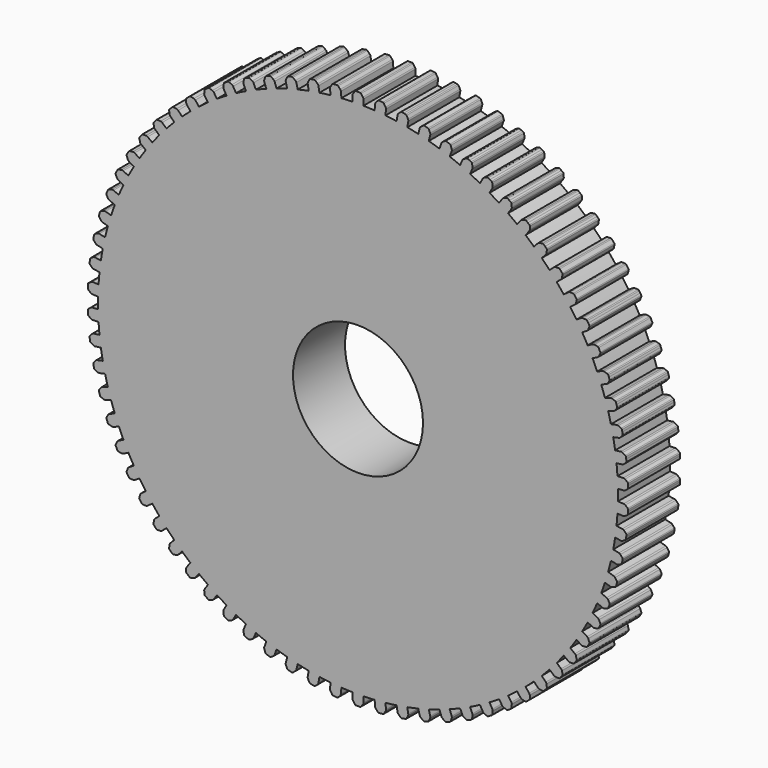
from build123d import *

# Parameters (mm, degrees)
F0_R     = 5
F1_DEPTH = 2.5


# Not quite as in the source:
# - ends of sketch curves that miss each other by under 0.0002 mm in the source are joined


with BuildPart() as f1:
    # F0 (on Front) → F1 (new body, symmetric)
    with BuildSketch(Plane.XZ):
        with BuildLine():
            ThreePointArc((19.9953867751, -0.4295436113), (19.9988466605, -0.2147841916), (20, 0))
            ThreePointArc((20, 0), (19.9988466605, 0.2147841916), (19.9953867751, 0.4295436113))
            ThreePointArc((19.9953867751, 0.4295436113), (19.9819793241, 0.8488240639), (19.9597810082, 1.2677310851))
            ThreePointArc((19.9597810082, 1.2677310851), (19.9279497709, 1.6961184895), (19.8869253221, 2.1237234363))
            ThreePointArc((19.8869253221, 2.1237234363), (19.8380087052, 2.5403563949), (19.7803645618, 2.9558717501))
            ThreePointArc((19.7803645618, 2.9558717501), (19.712318207, 3.3800164064), (19.6351781164, 3.8026017852))
            ThreePointArc((19.6351781164, 3.8026017852), (19.551104779, 4.2135853999), (19.4584301354, 4.6227152914))
            ThreePointArc((19.4584301354, 4.6227152914), (19.3546589387, 5.0395612277), (19.2419590025, 5.4540823011))
            ThreePointArc((19.2419590025, 5.4540823011), (19.1233346948, 5.8564554255), (18.996297274, 6.2562520631))
            ThreePointArc((18.996297274, 6.2562520631), (18.8575489092, 6.6627958948), (18.710101133, 7.066266029))
            ThreePointArc((18.710101133, 7.066266029), (18.5577805459, 7.4571295556), (18.3972956555, 7.8447123953))
            ThreePointArc((18.3972956555, 7.8447123953), (18.2245698078, 8.2380249649), (18.0434365561, 8.6275371483))
            ThreePointArc((18.0434365561, 8.6275371483), (17.858517163, 9.0040748964), (17.6657411002, 9.3766513949))
            ThreePointArc((17.6657411002, 9.3766513949), (17.4602822632, 9.7538988763), (17.2467686054, 10.1266466647))
            ThreePointArc((17.2467686054, 10.1266466647), (17.0305827547, 10.4861456711), (16.8069044754, 10.8410314064))
            ThreePointArc((16.8069044754, 10.8410314064), (16.5701929849, 11.1994957228), (16.3258372916, 11.5527934599))
            ThreePointArc((16.3258372916, 11.5527934599), (16.0799426073, 11.8926635261), (15.8269737188, 12.2273015381))
            ThreePointArc((15.8269737188, 12.2273015381), (15.5607150864, 12.5643999459), (15.2872779461, 12.8957021134))
            ThreePointArc((15.2872779461, 12.8957021134), (15.0134461051, 13.2134944678), (14.7330092539, 13.5254736821))
            ThreePointArc((14.7330092539, 13.5254736821), (14.4391218791, 13.8387773796), (14.1385734126, 14.1456969378))
            ThreePointArc((14.1385734126, 14.1456969378), (13.8387773796, 14.4391218791), (13.5328931197, 14.7261944783))
            ThreePointArc((13.5328931197, 14.7261944783), (13.2134944678, 15.0134461051), (12.8880001338, 15.2937716915))
            ThreePointArc((12.8880001338, 15.2937716915), (12.5643999459, 15.5607150864), (12.2352721804, 15.8208127058))
            ThreePointArc((12.2352721804, 15.8208127058), (11.8926635261, 16.0799426073), (11.5445685186, 16.3316544697))
            ThreePointArc((11.5445685186, 16.3316544697), (11.1994957228, 16.5701929849), (10.8494958247, 16.8014416152))
            ThreePointArc((10.8494958247, 16.8014416152), (10.4861456711, 17.0305827547), (10.1179580227, 17.2518673033))
            ThreePointArc((10.1179580227, 17.2518673033), (9.7538988763, 17.4602822632), (9.385548603, 17.6610157528))
            ThreePointArc((9.385548603, 17.6610157528), (9.0040748964, 17.858517163), (8.6184474075, 18.0477800376))
            ThreePointArc((8.6184474075, 18.0477800376), (8.2380249649, 18.2245698078), (7.8539782885, 18.3933418672))
            ThreePointArc((7.8539782885, 18.3933418672), (7.4571295556, 18.5577805459), (7.0568406811, 18.7136581031))
            ThreePointArc((7.0568406811, 18.7136581031), (6.6627958948, 18.8575489092), (6.2658198805, 18.9931435319))
            ThreePointArc((6.2658198805, 18.9931435319), (5.8564554255, 19.1233346948), (5.4443892559, 19.2447038333))
            ThreePointArc((5.4443892559, 19.2447038333), (5.0395612277, 19.3546589387), (4.6325160967, 19.4560991623))
            ThreePointArc((4.6325160967, 19.4560991623), (4.2135853999, 19.551104779), (3.7927108814, 19.6370910313))
            ThreePointArc((3.7927108814, 19.6370910313), (3.3800164064, 19.712318207), (2.9658349282, 19.7788731524))
            ThreePointArc((2.9658349282, 19.7788731524), (2.5403563949, 19.8380087052), (2.1137059381, 19.8879925384))
            ThreePointArc((2.1137059381, 19.8879925384), (1.6961184895, 19.9279497709), (1.2777848511, 19.9591399082))
            ThreePointArc((1.2777848511, 19.9591399082), (0.8497844269, 19.9819385053), (0.4213937304, 19.9955601903))
            ThreePointArc((0.4213937304, 19.9955601903), (0.4204327132, 19.99558042), (0.4194716951, 19.9956006036))
            ThreePointArc((0.4194716951, 19.9956006036), (0.3416806472, 19.9970811454), (0.2638844282, 19.9982590494))
            ThreePointArc((0.2638844282, 19.9982590494), (-0.0003038538, 19.9999999977), (-0.2644920828, 19.998251022))
            ThreePointArc((-0.2644920828, 19.998251022), (-0.3419844566, 19.997075952), (-0.4194716951, 19.9956006036))
            ThreePointArc((-0.4194716951, 19.9956006036), (-0.8488240639, 19.9819793241), (-1.2777848511, 19.9591399082))
            ThreePointArc((-1.2777848511, 19.9591399082), (-1.6961184895, 19.9279497709), (-2.1137059381, 19.8879925384))
            ThreePointArc((-2.1137059381, 19.8879925384), (-2.5403563949, 19.8380087052), (-2.9658349282, 19.7788731524))
            ThreePointArc((-2.9658349282, 19.7788731524), (-3.3800164064, 19.712318207), (-3.7927108814, 19.6370910313))
            ThreePointArc((-3.7927108814, 19.6370910313), (-4.2135853999, 19.551104779), (-4.6325160967, 19.4560991623))
            ThreePointArc((-4.6325160967, 19.4560991623), (-5.0395612277, 19.3546589387), (-5.4443892559, 19.2447038333))
            ThreePointArc((-5.4443892559, 19.2447038333), (-5.8564554255, 19.1233346948), (-6.2658198805, 18.9931435319))
            ThreePointArc((-6.2658198805, 18.9931435319), (-6.6627958948, 18.8575489092), (-7.0568406811, 18.7136581031))
            ThreePointArc((-7.0568406811, 18.7136581031), (-7.4571295556, 18.5577805459), (-7.8539782885, 18.3933418672))
            ThreePointArc((-7.8539782885, 18.3933418672), (-8.2380249649, 18.2245698078), (-8.6184474075, 18.0477800376))
            ThreePointArc((-8.6184474075, 18.0477800376), (-9.0040748964, 17.858517163), (-9.385548603, 17.6610157528))
            ThreePointArc((-9.385548603, 17.6610157528), (-9.7538988763, 17.4602822632), (-10.1179580227, 17.2518673033))
            ThreePointArc((-10.1179580227, 17.2518673033), (-10.4861456711, 17.0305827547), (-10.8494958247, 16.8014416152))
            ThreePointArc((-10.8494958247, 16.8014416152), (-11.1994957228, 16.5701929849), (-11.5445685186, 16.3316544697))
            ThreePointArc((-11.5445685186, 16.3316544697), (-11.8926635261, 16.0799426073), (-12.2352721804, 15.8208127058))
            ThreePointArc((-12.2352721804, 15.8208127058), (-12.5643999459, 15.5607150864), (-12.8880001338, 15.2937716915))
            ThreePointArc((-12.8880001338, 15.2937716915), (-13.2134944678, 15.0134461051), (-13.5328931197, 14.7261944783))
            ThreePointArc((-13.5328931197, 14.7261944783), (-13.8387773796, 14.4391218791), (-14.1385734126, 14.1456969378))
            ThreePointArc((-14.1385734126, 14.1456969378), (-14.4391218791, 13.8387773796), (-14.7330092539, 13.5254736821))
            ThreePointArc((-14.7330092539, 13.5254736821), (-15.0134461051, 13.2134944678), (-15.2872779461, 12.8957021134))
            ThreePointArc((-15.2872779461, 12.8957021134), (-15.5607150864, 12.5643999459), (-15.8269737188, 12.2273015381))
            ThreePointArc((-15.8269737188, 12.2273015381), (-16.0799426073, 11.8926635261), (-16.3258372916, 11.5527934599))
            ThreePointArc((-16.3258372916, 11.5527934599), (-16.5701929849, 11.1994957228), (-16.8069044754, 10.8410314064))
            ThreePointArc((-16.8069044754, 10.8410314064), (-17.0305827547, 10.4861456711), (-17.2467686054, 10.1266466647))
            ThreePointArc((-17.2467686054, 10.1266466647), (-17.4602822632, 9.7538988763), (-17.6657411002, 9.3766513949))
            ThreePointArc((-17.6657411002, 9.3766513949), (-17.858517163, 9.0040748964), (-18.0434365561, 8.6275371483))
            ThreePointArc((-18.0434365561, 8.6275371483), (-18.2245698078, 8.2380249649), (-18.3972956555, 7.8447123953))
            ThreePointArc((-18.3972956555, 7.8447123953), (-18.5577805459, 7.4571295556), (-18.710101133, 7.066266029))
            ThreePointArc((-18.710101133, 7.066266029), (-18.8575489092, 6.6627958948), (-18.996297274, 6.2562520631))
            ThreePointArc((-18.996297274, 6.2562520631), (-19.1233346948, 5.8564554255), (-19.2419590025, 5.4540823011))
            ThreePointArc((-19.2419590025, 5.4540823011), (-19.3546589387, 5.0395612277), (-19.4584301354, 4.6227152914))
            ThreePointArc((-19.4584301354, 4.6227152914), (-19.551104779, 4.2135853999), (-19.6351781164, 3.8026017852))
            ThreePointArc((-19.6351781164, 3.8026017852), (-19.712318207, 3.3800164064), (-19.7803645618, 2.9558717501))
            ThreePointArc((-19.7803645618, 2.9558717501), (-19.8380087052, 2.5403563949), (-19.8869253221, 2.1237234363))
            ThreePointArc((-19.8869253221, 2.1237234363), (-19.9279497709, 1.6961184895), (-19.9597810082, 1.2677310851))
            ThreePointArc((-19.9597810082, 1.2677310851), (-19.9819793241, 0.8488240639), (-19.9953867751, 0.4295436113))
            ThreePointArc((-19.9953867751, 0.4295436113), (-20, 0), (-19.9953867751, -0.4295436113))
            ThreePointArc((-19.9953867751, -0.4295436113), (-19.9819793241, -0.8488240639), (-19.9597810082, -1.2677310851))
            ThreePointArc((-19.9597810082, -1.2677310851), (-19.9279497709, -1.6961184895), (-19.8869253221, -2.1237234363))
            ThreePointArc((-19.8869253221, -2.1237234363), (-19.8380087052, -2.5403563949), (-19.7803645618, -2.9558717501))
            ThreePointArc((-19.7803645618, -2.9558717501), (-19.712318207, -3.3800164064), (-19.6351781164, -3.8026017852))
            ThreePointArc((-19.6351781164, -3.8026017852), (-19.551104779, -4.2135853999), (-19.4584301354, -4.6227152914))
            ThreePointArc((-19.4584301354, -4.6227152914), (-19.3546589387, -5.0395612277), (-19.2419590025, -5.4540823011))
            ThreePointArc((-19.2419590025, -5.4540823011), (-19.1233346948, -5.8564554255), (-18.996297274, -6.2562520631))
            ThreePointArc((-18.996297274, -6.2562520631), (-18.8575489092, -6.6627958948), (-18.710101133, -7.066266029))
            ThreePointArc((-18.710101133, -7.066266029), (-18.5577805459, -7.4571295556), (-18.3972956555, -7.8447123953))
            ThreePointArc((-18.3972956555, -7.8447123953), (-18.2245698078, -8.2380249649), (-18.0434365561, -8.6275371483))
            ThreePointArc((-18.0434365561, -8.6275371483), (-17.858517163, -9.0040748964), (-17.6657411002, -9.3766513949))
            ThreePointArc((-17.6657411002, -9.3766513949), (-17.4602822632, -9.7538988763), (-17.2467686054, -10.1266466647))
            ThreePointArc((-17.2467686054, -10.1266466647), (-17.0305827547, -10.4861456711), (-16.8069044754, -10.8410314064))
            ThreePointArc((-16.8069044754, -10.8410314064), (-16.5701929849, -11.1994957228), (-16.3258372916, -11.5527934599))
            ThreePointArc((-16.3258372916, -11.5527934599), (-16.0799426073, -11.8926635261), (-15.8269737188, -12.2273015381))
            ThreePointArc((-15.8269737188, -12.2273015381), (-15.5607150864, -12.5643999459), (-15.2872779461, -12.8957021134))
            ThreePointArc((-15.2872779461, -12.8957021134), (-15.0134461051, -13.2134944678), (-14.7330092539, -13.5254736821))
            ThreePointArc((-14.7330092539, -13.5254736821), (-14.4391218791, -13.8387773796), (-14.1385734126, -14.1456969378))
            ThreePointArc((-14.1385734126, -14.1456969378), (-13.8387773796, -14.4391218791), (-13.5328931197, -14.7261944783))
            ThreePointArc((-13.5328931197, -14.7261944783), (-13.2134944678, -15.0134461051), (-12.8880001338, -15.2937716915))
            ThreePointArc((-12.8880001338, -15.2937716915), (-12.5643999459, -15.5607150864), (-12.2352721804, -15.8208127058))
            ThreePointArc((-12.2352721804, -15.8208127058), (-11.8926635261, -16.0799426073), (-11.5445685186, -16.3316544697))
            ThreePointArc((-11.5445685186, -16.3316544697), (-11.1994957228, -16.5701929849), (-10.8494958247, -16.8014416152))
            ThreePointArc((-10.8494958247, -16.8014416152), (-10.4861456711, -17.0305827547), (-10.1179580227, -17.2518673033))
            ThreePointArc((-10.1179580227, -17.2518673033), (-9.7538988763, -17.4602822632), (-9.385548603, -17.6610157528))
            ThreePointArc((-9.385548603, -17.6610157528), (-9.0040748964, -17.858517163), (-8.6184474075, -18.0477800376))
            ThreePointArc((-8.6184474075, -18.0477800376), (-8.2380249649, -18.2245698078), (-7.8539782885, -18.3933418672))
            ThreePointArc((-7.8539782885, -18.3933418672), (-7.4580214618, -18.5574221236), (-7.0586394616, -18.7129796919))
            ThreePointArc((-7.0586394616, -18.7129796919), (-7.0577400795, -18.7133189192), (-7.0568406811, -18.7136581031))
            ThreePointArc((-7.0568406811, -18.7136581031), (-6.6627958948, -18.8575489092), (-6.2658198805, -18.9931435319))
            ThreePointArc((-6.2658198805, -18.9931435319), (-5.857374515, -19.1230532026), (-5.4462390896, -19.2441804133))
            ThreePointArc((-5.4462390896, -19.2441804133), (-5.4453141791, -19.2444421455), (-5.4443892559, -19.2447038333))
            ThreePointArc((-5.4443892559, -19.2447038333), (-5.0395612277, -19.3546589387), (-4.6325160967, -19.4560991623))
            ThreePointArc((-4.6325160967, -19.4560991623), (-4.2145250505, -19.5509022451), (-3.7945984401, -19.6367263738))
            ThreePointArc((-3.7945984401, -19.6367263738), (-3.7936546652, -19.6369087252), (-3.7927108814, -19.6370910313))
            ThreePointArc((-3.7927108814, -19.6370910313), (-3.3800164064, -19.712318207), (-2.9658349282, -19.7788731524))
            ThreePointArc((-2.9658349282, -19.7788731524), (-2.5413098365, -19.8378865889), (-2.115617622, -19.8877892707))
            ThreePointArc((-2.115617622, -19.8877892707), (-2.1146617825, -19.8878909275), (-2.1137059381, -19.8879925384))
            ThreePointArc((-2.1137059381, -19.8879925384), (-1.6961184895, -19.9279497709), (-1.2777848511, -19.9591399082))
            ThreePointArc((-1.2777848511, -19.9591399082), (-0.8497844269, -19.9819385053), (-0.4213937304, -19.9955601903))
            ThreePointArc((-0.4213937304, -19.9955601903), (-0.4204327132, -19.99558042), (-0.4194716951, -19.9956006036))
            ThreePointArc((-0.4194716951, -19.9956006036), (0, -20), (0.4194716951, -19.9956006036))
            ThreePointArc((0.4194716951, -19.9956006036), (0.847863699, -19.9820200968), (1.2758663127, -19.9592626405))
            ThreePointArc((1.2758663127, -19.9592626405), (1.2768255834, -19.9592012974), (1.2777848511, -19.9591399082))
            ThreePointArc((1.2777848511, -19.9591399082), (1.6961184895, -19.9279497709), (2.1137059381, -19.8879925384))
            ThreePointArc((2.1137059381, -19.8879925384), (2.5394029475, -19.8381307756), (2.9639337098, -19.779158146))
            ThreePointArc((2.9639337098, -19.779158146), (2.9648843224, -19.779015672), (2.9658349282, -19.7788731524))
            ThreePointArc((2.9658349282, -19.7788731524), (3.3800164064, -19.712318207), (3.7927108814, -19.6370910313))
            ThreePointArc((3.7927108814, -19.6370910313), (4.2126457396, -19.5513072676), (4.6306458965, -19.4565443638))
            ThreePointArc((4.6306458965, -19.4565443638), (4.631581002, -19.4563217855), (4.6325160967, -19.4560991623))
            ThreePointArc((4.6325160967, -19.4560991623), (5.0395612277, -19.3546589387), (5.4443892559, -19.2447038333))
            ThreePointArc((5.4443892559, -19.2447038333), (5.8555363225, -19.1236161428), (6.2639941735, -18.9937457336))
            ThreePointArc((6.2639941735, -18.9937457336), (6.2649070343, -18.9934446547), (6.2658198805, -18.9931435319))
            ThreePointArc((6.2658198805, -18.9931435319), (6.6627958948, -18.8575489092), (7.0568406811, -18.7136581031))
            ThreePointArc((7.0568406811, -18.7136581031), (7.4571295556, -18.5577805459), (7.8539782885, -18.3933418672))
            ThreePointArc((7.8539782885, -18.3933418672), (8.2380249649, -18.2245698078), (8.6184474075, -18.0477800376))
            ThreePointArc((8.6184474075, -18.0477800376), (9.0040748964, -17.858517163), (9.385548603, -17.6610157528))
            ThreePointArc((9.385548603, -17.6610157528), (9.7538988763, -17.4602822632), (10.1179580227, -17.2518673033))
            ThreePointArc((10.1179580227, -17.2518673033), (10.4861456711, -17.0305827547), (10.8494958247, -16.8014416152))
            ThreePointArc((10.8494958247, -16.8014416152), (11.1994957228, -16.5701929849), (11.5445685186, -16.3316544697))
            ThreePointArc((11.5445685186, -16.3316544697), (11.8926635261, -16.0799426073), (12.2352721804, -15.8208127058))
            ThreePointArc((12.2352721804, -15.8208127058), (12.5643999459, -15.5607150864), (12.8880001338, -15.2937716915))
            ThreePointArc((12.8880001338, -15.2937716915), (13.2134944678, -15.0134461051), (13.5328931197, -14.7261944783))
            ThreePointArc((13.5328931197, -14.7261944783), (13.8387773796, -14.4391218791), (14.1385734126, -14.1456969378))
            ThreePointArc((14.1385734126, -14.1456969378), (14.4391218791, -13.8387773796), (14.7330092539, -13.5254736821))
            ThreePointArc((14.7330092539, -13.5254736821), (15.0134461051, -13.2134944678), (15.2872779461, -12.8957021134))
            ThreePointArc((15.2872779461, -12.8957021134), (15.5607150864, -12.5643999459), (15.8269737188, -12.2273015381))
            ThreePointArc((15.8269737188, -12.2273015381), (16.0799426073, -11.8926635261), (16.3258372916, -11.5527934599))
            ThreePointArc((16.3258372916, -11.5527934599), (16.5701929849, -11.1994957228), (16.8069044754, -10.8410314064))
            ThreePointArc((16.8069044754, -10.8410314064), (17.0305827547, -10.4861456711), (17.2467686054, -10.1266466647))
            ThreePointArc((17.2467686054, -10.1266466647), (17.4602822632, -9.7538988763), (17.6657411002, -9.3766513949))
            ThreePointArc((17.6657411002, -9.3766513949), (17.858517163, -9.0040748964), (18.0434365561, -8.6275371483))
            ThreePointArc((18.0434365561, -8.6275371483), (18.2245698078, -8.2380249649), (18.3972956555, -7.8447123953))
            ThreePointArc((18.3972956555, -7.8447123953), (18.5577805459, -7.4571295556), (18.710101133, -7.066266029))
            ThreePointArc((18.710101133, -7.066266029), (18.8575489092, -6.6627958948), (18.996297274, -6.2562520631))
            ThreePointArc((18.996297274, -6.2562520631), (19.1233346948, -5.8564554255), (19.2419590025, -5.4540823011))
            ThreePointArc((19.2419590025, -5.4540823011), (19.3546589387, -5.0395612277), (19.4584301354, -4.6227152914))
            ThreePointArc((19.4584301354, -4.6227152914), (19.551104779, -4.2135853999), (19.6351781164, -3.8026017852))
            ThreePointArc((19.6351781164, -3.8026017852), (19.712318207, -3.3800164064), (19.7803645618, -2.9558717501))
            ThreePointArc((19.7803645618, -2.9558717501), (19.8380087052, -2.5403563949), (19.8869253221, -2.1237234363))
            ThreePointArc((19.8869253221, -2.1237234363), (19.9279497709, -1.6961184895), (19.9597810082, -1.2677310851))
            ThreePointArc((19.9597810082, -1.2677310851), (19.9819793241, -0.8488240639), (19.9953867751, -0.4295436113))
        make_face()
        Circle(F0_R, mode=Mode.SUBTRACT)
        with BuildLine():
            ThreePointArc((19.9597810082, 1.2677310851), (19.9819793241, 0.8488240639), (19.9953867751, 0.4295436113))
            Line((19.9953867751, 0.4295436113), (20.4440658139, 0.448603263))
            ThreePointArc((20.4440658139, 0.448603263), (20.5078544057, 0.4619396535), (20.5639692872, 0.4950751909))
            Line((20.5639692872, 0.4950751909), (20.7524823155, 0.6529092158))
            ThreePointArc((20.7524823155, 0.6529092158), (20.7797720171, 0.6892050283), (20.7881963552, 0.7338272688))
            Line((20.7881963552, 0.7338272688), (20.7818679474, 0.8828029156))
            Line((20.7818679474, 0.8828029156), (20.7755395396, 1.0317785625))
            ThreePointArc((20.7755395396, 1.0317785625), (20.7633613199, 1.075525617), (20.7330918299, 1.1093763451))
            Line((20.7330918299, 1.1093763451), (20.5318726614, 1.2506547495))
            ThreePointArc((20.5318726614, 1.2506547495), (20.4731498446, 1.2789120413), (20.4084600471, 1.2867907368))
            Line((20.4084600471, 1.2867907368), (19.9597810082, 1.2677310851))
        make_face()
        with BuildLine():
            Line((20.4440658139, -0.448603263), (19.9953867751, -0.4295436113))
            ThreePointArc((19.9953867751, -0.4295436113), (19.9819793241, -0.8488240639), (19.9597810082, -1.2677310851))
            Line((19.9597810082, -1.2677310851), (20.4084600471, -1.2867907368))
            ThreePointArc((20.4084600471, -1.2867907368), (20.4731498446, -1.2789120413), (20.5318726614, -1.2506547495))
            Line((20.5318726614, -1.2506547495), (20.7330918299, -1.1093763451))
            ThreePointArc((20.7330918299, -1.1093763451), (20.7633613199, -1.075525617), (20.7755395396, -1.0317785625))
            Line((20.7755395396, -1.0317785625), (20.7818679474, -0.8828029156))
            Line((20.7818679474, -0.8828029156), (20.7881963552, -0.7338272688))
            ThreePointArc((20.7881963552, -0.7338272688), (20.7797720171, -0.6892050283), (20.7524823155, -0.6529092158))
            Line((20.7524823155, -0.6529092158), (20.5639692872, -0.4950751909))
            ThreePointArc((20.5639692872, -0.4950751909), (20.5078544057, -0.4619396535), (20.4440658139, -0.448603263))
        make_face()
        with BuildLine():
            ThreePointArc((19.7803645618, 2.9558717501), (19.8380087052, 2.5403563949), (19.8869253221, 2.1237234363))
            Line((19.8869253221, 2.1237234363), (20.3323716182, 2.180765066))
            ThreePointArc((20.3323716182, 2.180765066), (20.3947994059, 2.1994630625), (20.447902043, 2.2372381031))
            Line((20.447902043, 2.2372381031), (20.6223506906, 2.4104905508))
            ThreePointArc((20.6223506906, 2.4104905508), (20.6464639808, 2.4489699356), (20.6510737398, 2.4941458577))
            Line((20.6510737398, 2.4941458577), (20.6321341127, 2.6420481316))
            Line((20.6321341127, 2.6420481316), (20.6131944855, 2.7899504055))
            ThreePointArc((20.6131944855, 2.7899504055), (20.5973501286, 2.8325070756), (20.5643189425, 2.863668824))
            Line((20.5643189425, 2.863668824), (20.3518434227, 2.9873736937))
            ThreePointArc((20.3518434227, 2.9873736937), (20.2909357698, 3.0105491455), (20.2258108579, 3.0129133798))
            Line((20.2258108579, 3.0129133798), (19.7803645618, 2.9558717501))
        make_face()
        with BuildLine():
            Line((20.3323716182, -2.180765066), (19.8869253221, -2.1237234363))
            ThreePointArc((19.8869253221, -2.1237234363), (19.8380087052, -2.5403563949), (19.7803645618, -2.9558717501))
            Line((19.7803645618, -2.9558717501), (20.2258108579, -3.0129133798))
            ThreePointArc((20.2258108579, -3.0129133798), (20.2909357698, -3.0105491455), (20.3518434227, -2.9873736937))
            Line((20.3518434227, -2.9873736937), (20.5643189425, -2.863668824))
            ThreePointArc((20.5643189425, -2.863668824), (20.5973501286, -2.8325070756), (20.6131944855, -2.7899504055))
            Line((20.6131944855, -2.7899504055), (20.6321341127, -2.6420481316))
            Line((20.6321341127, -2.6420481316), (20.6510737398, -2.4941458577))
            ThreePointArc((20.6510737398, -2.4941458577), (20.6464639808, -2.4489699356), (20.6223506906, -2.4104905508))
            Line((20.6223506906, -2.4104905508), (20.447902043, -2.2372381031))
            ThreePointArc((20.447902043, -2.2372381031), (20.3947994059, -2.1994630625), (20.3323716182, -2.180765066))
        make_face()
        with BuildLine():
            ThreePointArc((19.4584301354, 4.6227152914), (19.551104779, 4.2135853999), (19.6351781164, 3.8026017852))
            Line((19.6351781164, 3.8026017852), (20.074182219, 3.8972144067))
            ThreePointArc((20.074182219, 3.8972144067), (20.134799409, 3.9211392897), (20.184507196, 3.9632816635))
            Line((20.184507196, 3.9632816635), (20.3436345564, 4.1507042461))
            ThreePointArc((20.3436345564, 4.1507042461), (20.3643976983, 4.1910899584), (20.3651596648, 4.2364940686))
            Line((20.3651596648, 4.2364940686), (20.3337452788, 4.3822573303))
            Line((20.3337452788, 4.3822573303), (20.3023308929, 4.5280205919))
            ThreePointArc((20.3023308929, 4.5280205919), (20.2829345576, 4.5690802558), (20.2473796659, 4.5973285034))
            Line((20.2473796659, 4.5973285034), (20.0251786858, 4.7025685419))
            ThreePointArc((20.0251786858, 4.7025685419), (19.9625250377, 4.7204951741), (19.897434238, 4.7173279129))
            Line((19.897434238, 4.7173279129), (19.4584301354, 4.6227152914))
        make_face()
        with BuildLine():
            Line((20.074182219, -3.8972144067), (19.6351781164, -3.8026017852))
            ThreePointArc((19.6351781164, -3.8026017852), (19.551104779, -4.2135853999), (19.4584301354, -4.6227152914))
            Line((19.4584301354, -4.6227152914), (19.897434238, -4.7173279129))
            ThreePointArc((19.897434238, -4.7173279129), (19.9625250377, -4.7204951741), (20.0251786858, -4.7025685419))
            Line((20.0251786858, -4.7025685419), (20.2473796659, -4.5973285034))
            ThreePointArc((20.2473796659, -4.5973285034), (20.2829345576, -4.5690802558), (20.3023308929, -4.5280205919))
            Line((20.3023308929, -4.5280205919), (20.3337452788, -4.3822573303))
            Line((20.3337452788, -4.3822573303), (20.3651596648, -4.2364940686))
            ThreePointArc((20.3651596648, -4.2364940686), (20.3643976983, -4.1910899584), (20.3436345564, -4.1507042461))
            Line((20.3436345564, -4.1507042461), (20.184507196, -3.9632816635))
            ThreePointArc((20.184507196, -3.9632816635), (20.134799409, -3.9211392897), (20.074182219, -3.8972144067))
        make_face()
        with BuildLine():
            ThreePointArc((18.996297274, 6.2562520631), (19.1233346948, 5.8564554255), (19.2419590025, 5.4540823011))
            Line((19.2419590025, 5.4540823011), (19.6713578769, 5.5855842283))
            ThreePointArc((19.6713578769, 5.5855842283), (19.729727721, 5.6145636185), (19.7756825121, 5.6607696888))
            Line((19.7756825121, 5.6607696888), (19.918342069, 5.8610120222))
            ThreePointArc((19.918342069, 5.8610120222), (19.9356054638, 5.903013082), (19.9325141477, 5.9483182426))
            Line((19.9325141477, 5.9483182426), (19.8888513443, 6.0908922644))
            Line((19.8888513443, 6.0908922644), (19.8451885409, 6.2334662863))
            ThreePointArc((19.8451885409, 6.2334662863), (19.8223799784, 6.2727331081), (19.7845575548, 6.2978643255))
            Line((19.7845575548, 6.2978643255), (19.5542320775, 6.3838812761))
            ThreePointArc((19.5542320775, 6.3838812761), (19.4902838553, 6.3964299269), (19.4256961484, 6.3877539903))
            Line((19.4256961484, 6.3877539903), (18.996297274, 6.2562520631))
        make_face()
        with BuildLine():
            Line((19.6713578769, -5.5855842283), (19.2419590025, -5.4540823011))
            ThreePointArc((19.2419590025, -5.4540823011), (19.1233346948, -5.8564554255), (18.996297274, -6.2562520631))
            Line((18.996297274, -6.2562520631), (19.4256961484, -6.3877539903))
            ThreePointArc((19.4256961484, -6.3877539903), (19.4902838553, -6.3964299269), (19.5542320775, -6.3838812761))
            Line((19.5542320775, -6.3838812761), (19.7845575548, -6.2978643255))
            ThreePointArc((19.7845575548, -6.2978643255), (19.8223799784, -6.2727331081), (19.8451885409, -6.2334662863))
            Line((19.8451885409, -6.2334662863), (19.8888513443, -6.0908922644))
            Line((19.8888513443, -6.0908922644), (19.9325141477, -5.9483182426))
            ThreePointArc((19.9325141477, -5.9483182426), (19.9356054638, -5.903013082), (19.918342069, -5.8610120222))
            Line((19.918342069, -5.8610120222), (19.7756825121, -5.6607696888))
            ThreePointArc((19.7756825121, -5.6607696888), (19.729727721, -5.6145636185), (19.6713578769, -5.5855842283))
        make_face()
        with BuildLine():
            ThreePointArc((18.3972956555, 7.8447123953), (18.5577805459, 7.4571295556), (18.710101133, 7.066266029))
            Line((18.710101133, 7.066266029), (19.1268009505, 7.2337097876))
            ThreePointArc((19.1268009505, 7.2337097876), (19.1825028926, 7.2675348878), (19.2243735826, 7.3174717387))
            Line((19.2243735826, 7.3174717387), (19.3495374705, 7.5290910725))
            ThreePointArc((19.3495374705, 7.5290910725), (19.3631767351, 7.572404861), (19.3562544095, 7.6172846474))
            Line((19.3562544095, 7.6172846474), (19.3006577801, 7.7556421803))
            Line((19.3006577801, 7.7556421803), (19.2450611507, 7.8939997131))
            ThreePointArc((19.2450611507, 7.8939997131), (19.2190046972, 7.9311907746), (19.1791872532, 7.9530238909))
            Line((19.1791872532, 7.9530238909), (18.942396779, 8.0191979994))
            ThreePointArc((18.942396779, 8.0191979994), (18.8776147311, 8.0262782554), (18.813995473, 8.0121561538))
            Line((18.813995473, 8.0121561538), (18.3972956555, 7.8447123953))
        make_face()
        with BuildLine():
            Line((19.1268009505, -7.2337097876), (18.710101133, -7.066266029))
            ThreePointArc((18.710101133, -7.066266029), (18.5577805459, -7.4571295556), (18.3972956555, -7.8447123953))
            Line((18.3972956555, -7.8447123953), (18.813995473, -8.0121561538))
            ThreePointArc((18.813995473, -8.0121561538), (18.8776147311, -8.0262782554), (18.942396779, -8.0191979994))
            Line((18.942396779, -8.0191979994), (19.1791872532, -7.9530238909))
            ThreePointArc((19.1791872532, -7.9530238909), (19.2190046972, -7.9311907746), (19.2450611507, -7.8939997131))
            Line((19.2450611507, -7.8939997131), (19.3006577801, -7.7556421803))
            Line((19.3006577801, -7.7556421803), (19.3562544095, -7.6172846474))
            ThreePointArc((19.3562544095, -7.6172846474), (19.3631767351, -7.572404861), (19.3495374705, -7.5290910725))
            Line((19.3495374705, -7.5290910725), (19.2243735826, -7.3174717387))
            ThreePointArc((19.2243735826, -7.3174717387), (19.1825028926, -7.2675348878), (19.1268009505, -7.2337097876))
        make_face()
        with BuildLine():
            ThreePointArc((17.6657411002, 9.3766513949), (17.858517163, 9.0040748964), (18.0434365561, 8.6275371483))
            Line((18.0434365561, 8.6275371483), (18.444434985, 8.8297163021))
            ThreePointArc((18.444434985, 8.8297163021), (18.4970676913, 8.8681434016), (18.5345526008, 8.921451237))
            Line((18.5345526008, 8.921451237), (18.6413190112, 9.142922849))
            ThreePointArc((18.6413190112, 9.142922849), (18.6512358743, 9.1872372896), (18.6405324147, 9.2313683418))
            Line((18.6405324147, 9.2313683418), (18.5734025343, 9.3645125165))
            Line((18.5734025343, 9.3645125165), (18.5062726539, 9.4976566912))
            ThreePointArc((18.5062726539, 9.4976566912), (18.4771560468, 9.5325040298), (18.4356304679, 9.5508817369))
            Line((18.4356304679, 9.5508817369), (18.1940810777, 9.5967362174))
            ThreePointArc((18.1940810777, 9.5967362174), (18.1289319602, 9.5982970652), (18.0667395291, 9.5788305486))
            Line((18.0667395291, 9.5788305486), (17.6657411002, 9.3766513949))
        make_face()
        with BuildLine():
            Line((18.444434985, -8.8297163021), (18.0434365561, -8.6275371483))
            ThreePointArc((18.0434365561, -8.6275371483), (17.858517163, -9.0040748964), (17.6657411002, -9.3766513949))
            Line((17.6657411002, -9.3766513949), (18.0667395291, -9.5788305486))
            ThreePointArc((18.0667395291, -9.5788305486), (18.1289319602, -9.5982970652), (18.1940810777, -9.5967362174))
            Line((18.1940810777, -9.5967362174), (18.4356304679, -9.5508817369))
            ThreePointArc((18.4356304679, -9.5508817369), (18.4771560468, -9.5325040298), (18.5062726539, -9.4976566912))
            Line((18.5062726539, -9.4976566912), (18.5734025343, -9.3645125165))
            Line((18.5734025343, -9.3645125165), (18.6405324147, -9.2313683418))
            ThreePointArc((18.6405324147, -9.2313683418), (18.6512358743, -9.1872372896), (18.6413190112, -9.142922849))
            Line((18.6413190112, -9.142922849), (18.5345526008, -8.921451237))
            ThreePointArc((18.5345526008, -8.921451237), (18.4970676913, -8.8681434016), (18.444434985, -8.8297163021))
        make_face()
        with BuildLine():
            ThreePointArc((16.8069044754, 10.8410314064), (17.0305827547, 10.4861456711), (17.2467686054, 10.1266466647))
            Line((17.2467686054, 10.1266466647), (17.6291764428, 10.3621045083))
            ThreePointArc((17.6291764428, 10.3621045083), (17.6783606935, 10.4048567391), (17.7111897429, 10.4611514748))
            Line((17.7111897429, 10.4611514748), (17.7987894213, 10.6908796568))
            ThreePointArc((17.7987894213, 10.6908796568), (17.8049124317, 10.7358754629), (17.7905049567, 10.7789398157))
            Line((17.7905049567, 10.7789398157), (17.7123254976, 10.9059113254))
            Line((17.7123254976, 10.9059113254), (17.6341460386, 11.0328828352))
            ThreePointArc((17.6341460386, 11.0328828352), (17.6021790636, 11.065135375), (17.5592445427, 11.0799252611))
            Line((17.5592445427, 11.0799252611), (17.3146766053, 11.105129731))
            ThreePointArc((17.3146766053, 11.105129731), (17.2496298191, 11.1011599247), (17.1893123129, 11.0764892499))
            Line((17.1893123129, 11.0764892499), (16.8069044754, 10.8410314064))
        make_face()
        with BuildLine():
            Line((17.6291764428, -10.3621045083), (17.2467686054, -10.1266466647))
            ThreePointArc((17.2467686054, -10.1266466647), (17.0305827547, -10.4861456711), (16.8069044754, -10.8410314064))
            Line((16.8069044754, -10.8410314064), (17.1893123129, -11.0764892499))
            ThreePointArc((17.1893123129, -11.0764892499), (17.2496298191, -11.1011599247), (17.3146766053, -11.105129731))
            Line((17.3146766053, -11.105129731), (17.5592445427, -11.0799252611))
            ThreePointArc((17.5592445427, -11.0799252611), (17.6021790636, -11.065135375), (17.6341460386, -11.0328828352))
            Line((17.6341460386, -11.0328828352), (17.7123254976, -10.9059113254))
            Line((17.7123254976, -10.9059113254), (17.7905049567, -10.7789398157))
            ThreePointArc((17.7905049567, -10.7789398157), (17.8049124317, -10.7358754629), (17.7987894213, -10.6908796568))
            Line((17.7987894213, -10.6908796568), (17.7111897429, -10.4611514748))
            ThreePointArc((17.7111897429, -10.4611514748), (17.6783606935, -10.4048567391), (17.6291764428, -10.3621045083))
        make_face()
        with BuildLine():
            ThreePointArc((15.8269737188, 12.2273015381), (16.0799426073, 11.8926635261), (16.3258372916, 11.5527934599))
            Line((16.3258372916, 11.5527934599), (16.6868992804, 11.819833514))
            ThreePointArc((16.6868992804, 11.819833514), (16.7322807018, 11.8666028453), (16.760217357, 11.9254788765))
            Line((16.760217357, 11.9254788765), (16.8280191457, 12.1618084318))
            ThreePointArc((16.8280191457, 12.1618084318), (16.8303041869, 12.2071614075), (16.8122965028, 12.2488487813))
            Line((16.8122965028, 12.2488487813), (16.7236307499, 12.3687327934))
            Line((16.7236307499, 12.3687327934), (16.634964997, 12.4886168055))
            ThreePointArc((16.634964997, 12.4886168055), (16.6003779769, 12.5180421663), (16.5563438581, 12.52913767))
            Line((16.5563438581, 12.52913767), (16.3105194912, 12.5335105304))
            ThreePointArc((16.3105194912, 12.5335105304), (16.2460436999, 12.5240386725), (16.1880357076, 12.4943415922))
            Line((16.1880357076, 12.4943415922), (15.8269737188, 12.2273015381))
        make_face()
        with BuildLine():
            Line((16.6868992804, -11.819833514), (16.3258372916, -11.5527934599))
            ThreePointArc((16.3258372916, -11.5527934599), (16.0799426073, -11.8926635261), (15.8269737188, -12.2273015381))
            Line((15.8269737188, -12.2273015381), (16.1880357076, -12.4943415922))
            ThreePointArc((16.1880357076, -12.4943415922), (16.2460436999, -12.5240386725), (16.3105194912, -12.5335105304))
            Line((16.3105194912, -12.5335105304), (16.5563438581, -12.52913767))
            ThreePointArc((16.5563438581, -12.52913767), (16.6003779769, -12.5180421663), (16.634964997, -12.4886168055))
            Line((16.634964997, -12.4886168055), (16.7236307499, -12.3687327934))
            Line((16.7236307499, -12.3687327934), (16.8122965028, -12.2488487813))
            ThreePointArc((16.8122965028, -12.2488487813), (16.8303041869, -12.2071614075), (16.8280191457, -12.1618084318))
            Line((16.8280191457, -12.1618084318), (16.760217357, -11.9254788765))
            ThreePointArc((16.760217357, -11.9254788765), (16.7322807018, -11.8666028453), (16.6868992804, -11.819833514))
        make_face()
        with BuildLine():
            ThreePointArc((14.7330092539, 13.5254736821), (15.0134461051, 13.2134944678), (15.2872779461, 12.8957021134))
            Line((15.2872779461, 12.8957021134), (15.6243926262, 13.1924003485))
            ThreePointArc((15.6243926262, 13.1924003485), (15.6656442441, 13.2428498061), (15.6884872211, 13.3038829295))
            Line((15.6884872211, 13.3038829295), (15.7360026066, 13.5451110983))
            ThreePointArc((15.7360026066, 13.5451110983), (15.7344332149, 13.5904944745), (15.7129550674, 13.6305045107))
            Line((15.7129550674, 13.6305045107), (15.6144418594, 13.7424372581))
            Line((15.6144418594, 13.7424372581), (15.5159286514, 13.8543700055))
            ThreePointArc((15.5159286514, 13.8543700055), (15.4789707865, 13.880756177), (15.4341543367, 13.8880773548))
            Line((15.4341543367, 13.8880773548), (15.1888447104, 13.8715870992))
            ThreePointArc((15.1888447104, 13.8715870992), (15.1254044635, 13.8566814348), (15.070123934, 13.8221719171))
            Line((15.070123934, 13.8221719171), (14.7330092539, 13.5254736821))
        make_face()
        with BuildLine():
            Line((15.6243926262, -13.1924003485), (15.2872779461, -12.8957021134))
            ThreePointArc((15.2872779461, -12.8957021134), (15.0134461051, -13.2134944678), (14.7330092539, -13.5254736821))
            Line((14.7330092539, -13.5254736821), (15.070123934, -13.8221719171))
            ThreePointArc((15.070123934, -13.8221719171), (15.1254044635, -13.8566814348), (15.1888447104, -13.8715870992))
            Line((15.1888447104, -13.8715870992), (15.4341543367, -13.8880773548))
            ThreePointArc((15.4341543367, -13.8880773548), (15.4789707865, -13.880756177), (15.5159286514, -13.8543700055))
            Line((15.5159286514, -13.8543700055), (15.6144418594, -13.7424372581))
            Line((15.6144418594, -13.7424372581), (15.7129550674, -13.6305045107))
            ThreePointArc((15.7129550674, -13.6305045107), (15.7344332149, -13.5904944745), (15.7360026066, -13.5451110983))
            Line((15.7360026066, -13.5451110983), (15.6884872211, -13.3038829295))
            ThreePointArc((15.6884872211, -13.3038829295), (15.6656442441, -13.2428498061), (15.6243926262, -13.1924003485))
        make_face()
        with BuildLine():
            ThreePointArc((13.5328931197, 14.7261944783), (13.8387773796, 14.4391218791), (14.1385734126, 14.1456969378))
            Line((14.1385734126, 14.1456969378), (14.4493118652, 14.4699156361))
            ThreePointArc((14.4493118652, 14.4699156361), (14.4861364608, 14.5236817305), (14.5037211751, 14.5864322013))
            Line((14.5037211751, 14.5864322013), (14.5306078081, 14.830820929))
            ThreePointArc((14.5306078081, 14.830820929), (14.525195291, 14.8759077173), (14.5004014306, 14.9139521427))
            Line((14.5004014306, 14.9139521427), (14.3927505574, 15.0171271475))
            Line((14.3927505574, 15.0171271475), (14.2850996843, 15.1203021522))
            ThreePointArc((14.2850996843, 15.1203021522), (14.2460372569, 15.1434590213), (14.2007613796, 15.146953124))
            Line((14.2007613796, 15.146953124), (13.9577339554, 15.1097185652))
            ThreePointArc((13.9577339554, 15.1097185652), (13.8957863414, 15.0894864897), (13.8436315722, 15.0504131766))
            Line((13.8436315722, 15.0504131766), (13.5328931197, 14.7261944783))
        make_face()
        with BuildLine():
            Line((14.4493118652, -14.4699156361), (14.1385734126, -14.1456969378))
            ThreePointArc((14.1385734126, -14.1456969378), (13.8387773796, -14.4391218791), (13.5328931197, -14.7261944783))
            Line((13.5328931197, -14.7261944783), (13.8436315722, -15.0504131766))
            ThreePointArc((13.8436315722, -15.0504131766), (13.8957863414, -15.0894864897), (13.9577339554, -15.1097185652))
            Line((13.9577339554, -15.1097185652), (14.2007613796, -15.146953124))
            ThreePointArc((14.2007613796, -15.146953124), (14.2460372569, -15.1434590213), (14.2850996843, -15.1203021522))
            Line((14.2850996843, -15.1203021522), (14.3927505574, -15.0171271475))
            Line((14.3927505574, -15.0171271475), (14.5004014306, -14.9139521427))
            ThreePointArc((14.5004014306, -14.9139521427), (14.525195291, -14.8759077173), (14.5306078081, -14.830820929))
            Line((14.5306078081, -14.830820929), (14.5037211751, -14.5864322013))
            ThreePointArc((14.5037211751, -14.5864322013), (14.4861364608, -14.5236817305), (14.4493118652, -14.4699156361))
        make_face()
        with BuildLine():
            ThreePointArc((12.2352721804, 15.8208127058), (12.5643999459, 15.5607150864), (12.8880001338, 15.2937716915))
            Line((12.8880001338, 15.2937716915), (13.170123481, 15.64317485))
            ThreePointArc((13.170123481, 15.64317485), (13.2022557322, 15.6998701953), (13.2144554858, 15.7638858947))
            Line((13.2144554858, 15.7638858947), (13.2205196474, 16.009674355))
            ThreePointArc((13.2205196474, 16.009674355), (13.2113030021, 16.0541397041), (13.1833720693, 16.0899444078))
            Line((13.1833720693, 16.0899444078), (13.0673591579, 16.1836182916))
            Line((13.0673591579, 16.1836182916), (12.9513462466, 16.2772921754))
            ThreePointArc((12.9513462466, 16.2772921754), (12.9104607024, 16.2970528963), (12.8650516114, 16.2966947489))
            Line((12.8650516114, 16.2966947489), (12.6260574074, 16.2389841626))
            ThreePointArc((12.6260574074, 16.2389841626), (12.5660487603, 16.2135714488), (12.5173955276, 16.1702158643))
            Line((12.5173955276, 16.1702158643), (12.2352721804, 15.8208127058))
        make_face()
        with BuildLine():
            Line((13.170123481, -15.64317485), (12.8880001338, -15.2937716915))
            ThreePointArc((12.8880001338, -15.2937716915), (12.5643999459, -15.5607150864), (12.2352721804, -15.8208127058))
            Line((12.2352721804, -15.8208127058), (12.5173955276, -16.1702158643))
            ThreePointArc((12.5173955276, -16.1702158643), (12.5660487603, -16.2135714488), (12.6260574074, -16.2389841626))
            Line((12.6260574074, -16.2389841626), (12.8650516114, -16.2966947489))
            ThreePointArc((12.8650516114, -16.2966947489), (12.9104607024, -16.2970528963), (12.9513462466, -16.2772921754))
            Line((12.9513462466, -16.2772921754), (13.0673591579, -16.1836182916))
            Line((13.0673591579, -16.1836182916), (13.1833720693, -16.0899444078))
            ThreePointArc((13.1833720693, -16.0899444078), (13.2113030021, -16.0541397041), (13.2205196474, -16.009674355))
            Line((13.2205196474, -16.009674355), (13.2144554858, -15.7638858947))
            ThreePointArc((13.2144554858, -15.7638858947), (13.2022557322, -15.6998701953), (13.170123481, -15.64317485))
        make_face()
        with BuildLine():
            ThreePointArc((10.8494958247, 16.8014416152), (11.1994957228, 16.5701929849), (11.5445685186, 16.3316544697))
            Line((11.5445685186, 16.3316544697), (11.7960440554, 16.7037246306))
            ThreePointArc((11.7960440554, 16.7037246306), (11.8232524486, 16.7629407356), (11.8299793419, 16.8277604291))
            Line((11.8299793419, 16.8277604291), (11.8151773396, 17.0731777105))
            ThreePointArc((11.8151773396, 17.0731777105), (11.8022229724, 17.1167012465), (11.7713562101, 17.1500082548))
            Line((11.7713562101, 17.1500082548), (11.6478171363, 17.2335060952))
            Line((11.6478171363, 17.2335060952), (11.5242780625, 17.3170039355))
            ThreePointArc((11.5242780625, 17.3170039355), (11.4818639827, 17.3332261318), (11.4366488514, 17.3290183147))
            Line((11.4366488514, 17.3290183147), (11.2034098265, 17.251247507))
            ThreePointArc((11.2034098265, 17.251247507), (11.1457725099, 17.220837254), (11.1009713615, 17.1735117761))
            Line((11.1009713615, 17.1735117761), (10.8494958247, 16.8014416152))
        make_face()
        with BuildLine():
            Line((11.7960440554, -16.7037246306), (11.5445685186, -16.3316544697))
            ThreePointArc((11.5445685186, -16.3316544697), (11.1994957228, -16.5701929849), (10.8494958247, -16.8014416152))
            Line((10.8494958247, -16.8014416152), (11.1009713615, -17.1735117761))
            ThreePointArc((11.1009713615, -17.1735117761), (11.1457725099, -17.220837254), (11.2034098265, -17.251247507))
            Line((11.2034098265, -17.251247507), (11.4366488514, -17.3290183147))
            ThreePointArc((11.4366488514, -17.3290183147), (11.4818639827, -17.3332261318), (11.5242780625, -17.3170039355))
            Line((11.5242780625, -17.3170039355), (11.6478171363, -17.2335060952))
            Line((11.6478171363, -17.2335060952), (11.7713562101, -17.1500082548))
            ThreePointArc((11.7713562101, -17.1500082548), (11.8022229724, -17.1167012465), (11.8151773396, -17.0731777105))
            Line((11.8151773396, -17.0731777105), (11.8299793419, -16.8277604291))
            ThreePointArc((11.8299793419, -16.8277604291), (11.8232524486, -16.7629407356), (11.7960440554, -16.7037246306))
        make_face()
        with BuildLine():
            ThreePointArc((9.385548603, 17.6610157528), (9.7538988763, 17.4602822632), (10.1179580227, 17.2518673033))
            Line((10.1179580227, 17.2518673033), (10.3369738621, 17.6439236925))
            ThreePointArc((10.3369738621, 17.6439236925), (10.3590623602, 17.7052339038), (10.3602679257, 17.770390564))
            Line((10.3602679257, 17.770390564), (10.3247064084, 18.0136684293))
            ThreePointArc((10.3247064084, 18.0136684293), (10.3081076558, 18.0559365642), (10.2745274597, 18.0865058993))
            Line((10.2745274597, 18.0865058993), (10.1443523252, 18.1592260924))
            Line((10.1443523252, 18.1592260924), (10.0141771908, 18.2319462854))
            ThreePointArc((10.0141771908, 18.2319462854), (9.9705401699, 18.2445130758), (9.9258447745, 18.2364859064))
            Line((9.9258447745, 18.2364859064), (9.7000414211, 18.1392152178))
            ThreePointArc((9.7000414211, 18.1392152178), (9.6451907132, 18.1040265322), (9.6045644423, 18.053072142))
            Line((9.6045644423, 18.053072142), (9.385548603, 17.6610157528))
        make_face()
        with BuildLine():
            Line((10.3369738621, -17.6439236925), (10.1179580227, -17.2518673033))
            ThreePointArc((10.1179580227, -17.2518673033), (9.7538988763, -17.4602822632), (9.385548603, -17.6610157528))
            Line((9.385548603, -17.6610157528), (9.6045644423, -18.053072142))
            ThreePointArc((9.6045644423, -18.053072142), (9.6451907132, -18.1040265322), (9.7000414211, -18.1392152178))
            Line((9.7000414211, -18.1392152178), (9.9258447745, -18.2364859064))
            ThreePointArc((9.9258447745, -18.2364859064), (9.9705401699, -18.2445130758), (10.0141771908, -18.2319462854))
            Line((10.0141771908, -18.2319462854), (10.1443523252, -18.1592260924))
            Line((10.1443523252, -18.1592260924), (10.2745274597, -18.0865058993))
            ThreePointArc((10.2745274597, -18.0865058993), (10.3081076558, -18.0559365642), (10.3247064084, -18.0136684293))
            Line((10.3247064084, -18.0136684293), (10.3602679257, -17.770390564))
            ThreePointArc((10.3602679257, -17.770390564), (10.3590623602, -17.7052339038), (10.3369738621, -17.6439236925))
        make_face()
        with BuildLine():
            ThreePointArc((7.8539782885, 18.3933418672), (8.2380249649, 18.2245698078), (8.6184474075, 18.0477800376))
            Line((8.6184474075, 18.0477800376), (8.8034255352, 18.4569978799))
            ThreePointArc((8.8034255352, 18.4569978799), (8.8202349901, 18.5199604559), (8.8159105417, 18.5849846276))
            Line((8.8159105417, 18.5849846276), (8.7598457309, 18.8243702543))
            ThreePointArc((8.7598457309, 18.8243702543), (8.7397221872, 18.8650784452), (8.7036705034, 18.8926898543))
            Line((8.7036705034, 18.8926898543), (8.5677972232, 18.9541084495))
            Line((8.5677972232, 18.9541084495), (8.431923943, 19.0155270446))
            ThreePointArc((8.431923943, 19.0155270446), (8.3873783867, 19.0243478851), (8.3435247585, 19.0125591993))
            Line((8.3435247585, 19.0125591993), (8.1267839949, 18.8964894673))
            ThreePointArc((8.1267839949, 18.8964894673), (8.0751150963, 18.8567758843), (8.0389564162, 18.8025597095))
            Line((8.0389564162, 18.8025597095), (7.8539782885, 18.3933418672))
        make_face()
        with BuildLine():
            Line((8.8034255352, -18.4569978799), (8.6184474075, -18.0477800376))
            ThreePointArc((8.6184474075, -18.0477800376), (8.2380249649, -18.2245698078), (7.8539782885, -18.3933418672))
            Line((7.8539782885, -18.3933418672), (8.0389564162, -18.8025597095))
            ThreePointArc((8.0389564162, -18.8025597095), (8.0751150963, -18.8567758843), (8.1267839949, -18.8964894673))
            Line((8.1267839949, -18.8964894673), (8.3435247585, -19.0125591993))
            ThreePointArc((8.3435247585, -19.0125591993), (8.3869336837, -19.0243319643), (8.4311113506, -19.0158900135))
            Line((8.4311113506, -19.0158900135), (8.431923943, -19.0155270446))
            Line((8.431923943, -19.0155270446), (8.5669862299, -18.9544750416))
            Line((8.5669862299, -18.9544750416), (8.5677972232, -18.9541084495))
            Line((8.5677972232, -18.9541084495), (8.7036705034, -18.8926898543))
            ThreePointArc((8.7036705034, -18.8926898543), (8.7397221872, -18.8650784452), (8.7598457309, -18.8243702543))
            Line((8.7598457309, -18.8243702543), (8.8159105417, -18.5849846276))
            ThreePointArc((8.8159105417, -18.5849846276), (8.8202349901, -18.5199604559), (8.8034255352, -18.4569978799))
        make_face()
        with BuildLine():
            ThreePointArc((6.2658198805, 18.9931435319), (6.6627958948, 18.8575489092), (7.0568406811, 18.7136581031))
            Line((7.0568406811, 18.7136581031), (7.2064483256, 19.1370889746))
            ThreePointArc((7.2064483256, 19.1370889746), (7.2178576248, 19.2012502686), (7.2080343203, 19.2656734511))
            Line((7.2080343203, 19.2656734511), (7.1318701642, 19.4994420603))
            ThreePointArc((7.1318701642, 19.4994420603), (7.1083668201, 19.5382970037), (7.0701034018, 19.562751546))
            Line((7.0701034018, 19.562751546), (6.9295109459, 19.6124260208))
            Line((6.9295109459, 19.6124260208), (6.78891849, 19.6621004956))
            ThreePointArc((6.78891849, 19.6621004956), (6.74378535, 19.6671118319), (6.7010894554, 19.6516465674))
            Line((6.7010894554, 19.6516465674), (6.4949729038, 19.5176140772))
            ThreePointArc((6.4949729038, 19.5176140772), (6.4468580902, 19.4736617341), (6.415427525, 19.4165744034))
            Line((6.415427525, 19.4165744034), (6.2658198805, 18.9931435319))
        make_face()
        with BuildLine():
            Line((7.2064483256, -19.1370889746), (7.0568406811, -18.7136581031))
            ThreePointArc((7.0568406811, -18.7136581031), (6.6627958948, -18.8575489092), (6.2658198805, -18.9931435319))
            Line((6.2658198805, -18.9931435319), (6.415427525, -19.4165744034))
            ThreePointArc((6.415427525, -19.4165744034), (6.4468580902, -19.4736617341), (6.4949729038, -19.5176140772))
            Line((6.4949729038, -19.5176140772), (6.7010894554, -19.6516465674))
            ThreePointArc((6.7010894554, -19.6516465674), (6.7433435992, -19.667058255), (6.788078043, -19.6623932443))
            Line((6.788078043, -19.6623932443), (6.78891849, -19.6621004956))
            Line((6.78891849, -19.6621004956), (6.928671785, -19.6127225152))
            Line((6.928671785, -19.6127225152), (6.9295109459, -19.6124260208))
            Line((6.9295109459, -19.6124260208), (7.0701034018, -19.562751546))
            ThreePointArc((7.0701034018, -19.562751546), (7.1083668201, -19.5382970037), (7.1318701642, -19.4994420603))
            Line((7.1318701642, -19.4994420603), (7.2080343203, -19.2656734511))
            ThreePointArc((7.2080343203, -19.2656734511), (7.2178576248, -19.2012502686), (7.2064483256, -19.1370889746))
        make_face()
        with BuildLine():
            ThreePointArc((4.6325160967, 19.4560991623), (5.0395612277, 19.3546589387), (5.4443892559, 19.2447038333))
            Line((5.4443892559, 19.2447038333), (5.5575484906, 19.6792969048))
            ThreePointArc((5.5575484906, 19.6792969048), (5.5634754299, 19.7441946331), (5.5482240464, 19.807552656))
            Line((5.5482240464, 19.807552656), (5.4525093096, 20.0340199393))
            ThreePointArc((5.4525093096, 20.0340199393), (5.4257955071, 20.0707416846), (5.3855960431, 20.0918631646))
            Line((5.3855960431, 20.0918631646), (5.2412973834, 20.1294356133))
            Line((5.2412973834, 20.1294356133), (5.0969987237, 20.167008062))
            ThreePointArc((5.0969987237, 20.167008062), (5.0516031854, 20.1681737872), (5.0103726493, 20.1491433718))
            Line((5.0103726493, 20.1491433718), (4.8163653841, 19.9981138304))
            ThreePointArc((4.8163653841, 19.9981138304), (4.7721513237, 19.9502394049), (4.7456753314, 19.8906922338))
            Line((4.7456753314, 19.8906922338), (4.6325160967, 19.4560991623))
        make_face()
        with BuildLine():
            Line((5.5575484906, -19.6792969048), (5.4443892559, -19.2447038333))
            ThreePointArc((5.4443892559, -19.2447038333), (5.0395612277, -19.3546589387), (4.6325160967, -19.4560991623))
            Line((4.6325160967, -19.4560991623), (4.7456753314, -19.8906922338))
            ThreePointArc((4.7456753314, -19.8906922338), (4.7721513237, -19.9502394049), (4.8163653841, -19.9981138304))
            Line((4.8163653841, -19.9981138304), (5.0103726493, -20.1491433718))
            ThreePointArc((5.0103726493, -20.1491433718), (5.0511675696, -20.1680829403), (5.0961364776, -20.1672284812))
            Line((5.0961364776, -20.1672284812), (5.0969987237, -20.167008062))
            Line((5.0969987237, -20.167008062), (5.2404361011, -20.1296598738))
            Line((5.2404361011, -20.1296598738), (5.2412973834, -20.1294356133))
            Line((5.2412973834, -20.1294356133), (5.3855960431, -20.0918631646))
            ThreePointArc((5.3855960431, -20.0918631646), (5.4257955071, -20.0707416846), (5.4525093096, -20.0340199393))
            Line((5.4525093096, -20.0340199393), (5.5482240464, -19.807552656))
            ThreePointArc((5.5482240464, -19.807552656), (5.5634754299, -19.7441946331), (5.5575484906, -19.6792969048))
        make_face()
        with BuildLine():
            ThreePointArc((2.9658349282, 19.7788731524), (3.3800164064, 19.712318207), (3.7927108814, 19.6370910313))
            Line((3.7927108814, 19.6370910313), (3.8686063915, 20.0797150498))
            ThreePointArc((3.8686063915, 20.0797150498), (3.869008267, 20.1448816229), (3.8484386911, 20.20671799))
            Line((3.8484386911, 20.20671799), (3.7338630004, 20.4242522457))
            ThreePointArc((3.7338630004, 20.4242522457), (3.7041312131, 20.4585762117), (3.6622853416, 20.4762124486))
            Line((3.6622853416, 20.4762124486), (3.5153201532, 20.5014121609))
            Line((3.5153201532, 20.5014121609), (3.3683549648, 20.5266118733))
            ThreePointArc((3.3683549648, 20.5266118733), (3.323024104, 20.5239235883), (3.2835559934, 20.5014651364))
            Line((3.2835559934, 20.5014651364), (3.1030558415, 20.3345267152))
            ThreePointArc((3.1030558415, 20.3345267152), (3.0630610977, 20.2830751436), (3.0417304383, 20.2214971709))
            Line((3.0417304383, 20.2214971709), (2.9658349282, 19.7788731524))
        make_face()
        with BuildLine():
            ThreePointArc((1.2777848511, 19.9591399082), (1.6961184895, 19.9279497709), (2.1137059381, 19.8879925384))
            Line((2.1137059381, 19.8879925384), (2.1517908946, 20.3354583877))
            ThreePointArc((2.1517908946, 20.3354583877), (2.1466648109, 20.4004242789), (2.1209252469, 20.4602934579))
            Line((2.1209252469, 20.4602934579), (1.9883141228, 20.6673273466))
            ThreePointArc((1.9883141228, 20.6673273466), (1.9557785689, 20.6990062284), (1.9125877902, 20.7130301528))
            Line((1.9125877902, 20.7130301528), (1.7640149607, 20.7256755642))
            Line((1.7640149607, 20.7256755642), (1.6154421312, 20.7383209756))
            ThreePointArc((1.6154421312, 20.7383209756), (1.5705025578, 20.7317980496), (1.5330812413, 20.7060733749))
            Line((1.5330812413, 20.7060733749), (1.3673887104, 20.5244288691))
            ThreePointArc((1.3673887104, 20.5244288691), (1.3319014462, 20.4697708611), (1.3158698077, 20.4066057575))
            Line((1.3158698077, 20.4066057575), (1.2777848511, 19.9591399082))
        make_face()
        with BuildLine():
            Line((3.8686063915, -20.0797150498), (3.7927108814, -19.6370910313))
            ThreePointArc((3.7927108814, -19.6370910313), (3.3800164064, -19.712318207), (2.9658349282, -19.7788731524))
            Line((2.9658349282, -19.7788731524), (3.0417304383, -20.2214971709))
            ThreePointArc((3.0417304383, -20.2214971709), (3.0630610977, -20.2830751436), (3.1030558415, -20.3345267152))
            Line((3.1030558415, -20.3345267152), (3.2835559934, -20.5014651364))
            ThreePointArc((3.2835559934, -20.5014651364), (3.3225977619, -20.5237961259), (3.3674771321, -20.5267583747))
            Line((3.3674771321, -20.5267583747), (3.3683549648, -20.5266118733))
            Line((3.3683549648, -20.5266118733), (3.514442955, -20.5015625717))
            Line((3.514442955, -20.5015625717), (3.5153201532, -20.5014121609))
            Line((3.5153201532, -20.5014121609), (3.6622853416, -20.4762124486))
            ThreePointArc((3.6622853416, -20.4762124486), (3.7041312131, -20.4585762117), (3.7338630004, -20.4242522457))
            Line((3.7338630004, -20.4242522457), (3.8484386911, -20.20671799))
            ThreePointArc((3.8484386911, -20.20671799), (3.869008267, -20.1448816229), (3.8686063915, -20.0797150498))
        make_face()
        with BuildLine():
            ThreePointArc((0.2638844282, 19.9982590494), (0.3416806472, 19.9970811454), (0.4194716951, 19.9956006036))
            Line((0.4194716951, 19.9956006036), (0.4194716951, 20.444684282))
            ThreePointArc((0.4194716951, 20.444684282), (0.4088545857, 20.5089814105), (0.3781304876, 20.5664520426))
            Line((0.3781304876, 20.5664520426), (0.2284393963, 20.7614938803))
            ThreePointArc((0.2284393963, 20.7614938803), (0.1933344953, 20.7902994309), (0.14911, 20.80061))
            Line((0.14911, 20.80061), (0, 20.80061))
            Line((0, 20.80061), (0, 20.00061))
            add(Edge.make_bspline(
                [(0, 20.00061), (0.0878540401, 20.0006084582), (0.1758899381, 19.9996186426), (0.2638844282, 19.9982590494)],
                knots=[0.4994284917, 0.4994284917, 0.4994284917, 0.4994284917, 0.8128711967, 0.8128711967, 0.8128711967, 0.8128711967], degree=3))
        make_face()
        with BuildLine():
            Line((2.1517908946, -20.3354583877), (2.1137059381, -19.8879925384))
            ThreePointArc((2.1137059381, -19.8879925384), (1.6961184895, -19.9279497709), (1.2777848511, -19.9591399082))
            Line((1.2777848511, -19.9591399082), (1.3158698077, -20.4066057575))
            ThreePointArc((1.3158698077, -20.4066057575), (1.3319014462, -20.4697708611), (1.3673887104, -20.5244288691))
            Line((1.3673887104, -20.5244288691), (1.5330812413, -20.7060733749))
            ThreePointArc((1.5330812413, -20.7060733749), (1.5700885612, -20.73163489), (1.6145550367, -20.7383925038))
            Line((1.6145550367, -20.7383925038), (1.6154421312, -20.7383209756))
            Line((1.6154421312, -20.7383209756), (1.7631281669, -20.7257510414))
            Line((1.7631281669, -20.7257510414), (1.7640149607, -20.7256755642))
            Line((1.7640149607, -20.7256755642), (1.9125877902, -20.7130301528))
            ThreePointArc((1.9125877902, -20.7130301528), (1.9557785689, -20.6990062284), (1.9883141228, -20.6673273466))
            Line((1.9883141228, -20.6673273466), (2.1209252469, -20.4602934579))
            ThreePointArc((2.1209252469, -20.4602934579), (2.1466648109, -20.4004242789), (2.1517908946, -20.3354583877))
        make_face()
        with BuildLine():
            ThreePointArc((-0.4194716951, 19.9956006036), (-0.3419844566, 19.997075952), (-0.2644920828, 19.998251022))
            add(Edge.make_bspline(
                [(-0.2644920828, 19.998251022), (-0.176360151, 19.9996154015), (-0.0882718715, 20.0006115491), (0, 20.00061)],
                knots=[0.1844950618, 0.1844950618, 0.1844950618, 0.1844950618, 0.4994284917, 0.4994284917, 0.4994284917, 0.4994284917], degree=3))
            Line((0, 20.00061), (0, 20.80061))
            Line((0, 20.80061), (-0.14911, 20.80061))
            ThreePointArc((-0.14911, 20.80061), (-0.1933344953, 20.7902994309), (-0.2284393963, 20.7614938803))
            Line((-0.2284393963, 20.7614938803), (-0.3781304876, 20.5664520426))
            ThreePointArc((-0.3781304876, 20.5664520426), (-0.4088545857, 20.5089814105), (-0.4194716951, 20.444684282))
            Line((-0.4194716951, 20.444684282), (-0.4194716951, 19.9956006036))
        make_face()
        with BuildLine():
            Line((0.4194716951, -20.444684282), (0.4194716951, -19.9956006036))
            ThreePointArc((0.4194716951, -19.9956006036), (0, -20), (-0.4194716951, -19.9956006036))
            Line((-0.4194716951, -19.9956006036), (-0.4194716951, -20.444684282))
            ThreePointArc((-0.4194716951, -20.444684282), (-0.4088545857, -20.5089814105), (-0.3781304876, -20.5664520426))
            Line((-0.3781304876, -20.5664520426), (-0.2284393963, -20.7614938803))
            ThreePointArc((-0.2284393963, -20.7614938803), (-0.1937331635, -20.7901017498), (-0.1499999648, -20.8006060397))
            Line((-0.1499999648, -20.8006060397), (-0.14911, -20.80061))
            Line((-0.14911, -20.80061), (-0.00089, -20.80061))
            Line((-0.00089, -20.80061), (0, -20.80061))
            Line((0, -20.80061), (0.14911, -20.80061))
            ThreePointArc((0.14911, -20.80061), (0.1933344953, -20.7902994309), (0.2284393963, -20.7614938803))
            Line((0.2284393963, -20.7614938803), (0.3781304876, -20.5664520426))
            ThreePointArc((0.3781304876, -20.5664520426), (0.4088545857, -20.5089814105), (0.4194716951, -20.444684282))
        make_face()
        with BuildLine():
            ThreePointArc((-2.1137059381, 19.8879925384), (-1.6961184895, 19.9279497709), (-1.2777848511, 19.9591399082))
            Line((-1.2777848511, 19.9591399082), (-1.3158698077, 20.4066057575))
            ThreePointArc((-1.3158698077, 20.4066057575), (-1.3319014462, 20.4697708611), (-1.3673887104, 20.5244288691))
            Line((-1.3673887104, 20.5244288691), (-1.5330812413, 20.7060733749))
            ThreePointArc((-1.5330812413, 20.7060733749), (-1.5705025578, 20.7317980496), (-1.6154421312, 20.7383209756))
            Line((-1.6154421312, 20.7383209756), (-1.7640149607, 20.7256755642))
            Line((-1.7640149607, 20.7256755642), (-1.9125877902, 20.7130301528))
            ThreePointArc((-1.9125877902, 20.7130301528), (-1.9557785689, 20.6990062284), (-1.9883141228, 20.6673273466))
            Line((-1.9883141228, 20.6673273466), (-2.1209252469, 20.4602934579))
            ThreePointArc((-2.1209252469, 20.4602934579), (-2.1466648109, 20.4004242789), (-2.1517908946, 20.3354583877))
            Line((-2.1517908946, 20.3354583877), (-2.1137059381, 19.8879925384))
        make_face()
        with BuildLine():
            ThreePointArc((-3.7927108814, 19.6370910313), (-3.3800164064, 19.712318207), (-2.9658349282, 19.7788731524))
            Line((-2.9658349282, 19.7788731524), (-3.0417304383, 20.2214971709))
            ThreePointArc((-3.0417304383, 20.2214971709), (-3.0630610977, 20.2830751436), (-3.1030558415, 20.3345267152))
            Line((-3.1030558415, 20.3345267152), (-3.2835559934, 20.5014651364))
            ThreePointArc((-3.2835559934, 20.5014651364), (-3.323024104, 20.5239235883), (-3.3683549648, 20.5266118733))
            Line((-3.3683549648, 20.5266118733), (-3.5153201532, 20.5014121609))
            Line((-3.5153201532, 20.5014121609), (-3.6622853416, 20.4762124486))
            ThreePointArc((-3.6622853416, 20.4762124486), (-3.7041312131, 20.4585762117), (-3.7338630004, 20.4242522457))
            Line((-3.7338630004, 20.4242522457), (-3.8484386911, 20.20671799))
            ThreePointArc((-3.8484386911, 20.20671799), (-3.869008267, 20.1448816229), (-3.8686063915, 20.0797150498))
            Line((-3.8686063915, 20.0797150498), (-3.7927108814, 19.6370910313))
        make_face()
        with BuildLine():
            Line((-1.3158698077, -20.4066057575), (-1.2777848511, -19.9591399082))
            ThreePointArc((-1.2777848511, -19.9591399082), (-1.6961184895, -19.9279497709), (-2.1137059381, -19.8879925384))
            Line((-2.1137059381, -19.8879925384), (-2.1517908946, -20.3354583877))
            ThreePointArc((-2.1517908946, -20.3354583877), (-2.1466648109, -20.4004242789), (-2.1209252469, -20.4602934579))
            Line((-2.1209252469, -20.4602934579), (-1.9883141228, -20.6673273466))
            ThreePointArc((-1.9883141228, -20.6673273466), (-1.9561590364, -20.69877545), (-1.913474213, -20.7129507325))
            Line((-1.913474213, -20.7129507325), (-1.9125877902, -20.7130301528))
            Line((-1.9125877902, -20.7130301528), (-1.7649017545, -20.7256000869))
            Line((-1.7649017545, -20.7256000869), (-1.7640149607, -20.7256755642))
            Line((-1.7640149607, -20.7256755642), (-1.6154421312, -20.7383209756))
            ThreePointArc((-1.6154421312, -20.7383209756), (-1.5705025578, -20.7317980496), (-1.5330812413, -20.7060733749))
            Line((-1.5330812413, -20.7060733749), (-1.3673887104, -20.5244288691))
            ThreePointArc((-1.3673887104, -20.5244288691), (-1.3319014462, -20.4697708611), (-1.3158698077, -20.4066057575))
        make_face()
        with BuildLine():
            ThreePointArc((-5.4443892559, 19.2447038333), (-5.0395612277, 19.3546589387), (-4.6325160967, 19.4560991623))
            Line((-4.6325160967, 19.4560991623), (-4.7456753314, 19.8906922338))
            ThreePointArc((-4.7456753314, 19.8906922338), (-4.7721513237, 19.9502394049), (-4.8163653841, 19.9981138304))
            Line((-4.8163653841, 19.9981138304), (-5.0103726493, 20.1491433718))
            ThreePointArc((-5.0103726493, 20.1491433718), (-5.0516031854, 20.1681737872), (-5.0969987237, 20.167008062))
            Line((-5.0969987237, 20.167008062), (-5.2412973834, 20.1294356133))
            Line((-5.2412973834, 20.1294356133), (-5.3855960431, 20.0918631646))
            ThreePointArc((-5.3855960431, 20.0918631646), (-5.4257955071, 20.0707416846), (-5.4525093096, 20.0340199393))
            Line((-5.4525093096, 20.0340199393), (-5.5482240464, 19.807552656))
            ThreePointArc((-5.5482240464, 19.807552656), (-5.5634754299, 19.7441946331), (-5.5575484906, 19.6792969048))
            Line((-5.5575484906, 19.6792969048), (-5.4443892559, 19.2447038333))
        make_face()
        with BuildLine():
            Line((-3.0417304383, -20.2214971709), (-2.9658349282, -19.7788731524))
            ThreePointArc((-2.9658349282, -19.7788731524), (-3.3800164064, -19.712318207), (-3.7927108814, -19.6370910313))
            Line((-3.7927108814, -19.6370910313), (-3.8686063915, -20.0797150498))
            ThreePointArc((-3.8686063915, -20.0797150498), (-3.869008267, -20.1448816229), (-3.8484386911, -20.20671799))
            Line((-3.8484386911, -20.20671799), (-3.7338630004, -20.4242522457))
            ThreePointArc((-3.7338630004, -20.4242522457), (-3.7044907386, -20.4583139988), (-3.6631618357, -20.4760581405))
            Line((-3.6631618357, -20.4760581405), (-3.6622853416, -20.4762124486))
            Line((-3.6622853416, -20.4762124486), (-3.5161973514, -20.5012617502))
            Line((-3.5161973514, -20.5012617502), (-3.5153201532, -20.5014121609))
            Line((-3.5153201532, -20.5014121609), (-3.3683549648, -20.5266118733))
            ThreePointArc((-3.3683549648, -20.5266118733), (-3.323024104, -20.5239235883), (-3.2835559934, -20.5014651364))
            Line((-3.2835559934, -20.5014651364), (-3.1030558415, -20.3345267152))
            ThreePointArc((-3.1030558415, -20.3345267152), (-3.0630610977, -20.2830751436), (-3.0417304383, -20.2214971709))
        make_face()
        with BuildLine():
            ThreePointArc((-7.0568406811, 18.7136581031), (-6.6627958948, 18.8575489092), (-6.2658198805, 18.9931435319))
            Line((-6.2658198805, 18.9931435319), (-6.415427525, 19.4165744034))
            ThreePointArc((-6.415427525, 19.4165744034), (-6.4468580902, 19.4736617341), (-6.4949729038, 19.5176140772))
            Line((-6.4949729038, 19.5176140772), (-6.7010894554, 19.6516465674))
            ThreePointArc((-6.7010894554, 19.6516465674), (-6.74378535, 19.6671118319), (-6.78891849, 19.6621004956))
            Line((-6.78891849, 19.6621004956), (-6.9295109459, 19.6124260208))
            Line((-6.9295109459, 19.6124260208), (-7.0701034018, 19.562751546))
            ThreePointArc((-7.0701034018, 19.562751546), (-7.1083668201, 19.5382970037), (-7.1318701642, 19.4994420603))
            Line((-7.1318701642, 19.4994420603), (-7.2080343203, 19.2656734511))
            ThreePointArc((-7.2080343203, 19.2656734511), (-7.2178576248, 19.2012502686), (-7.2064483256, 19.1370889746))
            Line((-7.2064483256, 19.1370889746), (-7.0568406811, 18.7136581031))
        make_face()
        with BuildLine():
            ThreePointArc((-8.6184474075, 18.0477800376), (-8.2380249649, 18.2245698078), (-7.8539782885, 18.3933418672))
            Line((-7.8539782885, 18.3933418672), (-8.0389564162, 18.8025597095))
            ThreePointArc((-8.0389564162, 18.8025597095), (-8.0751150963, 18.8567758843), (-8.1267839949, 18.8964894673))
            Line((-8.1267839949, 18.8964894673), (-8.3435247585, 19.0125591993))
            ThreePointArc((-8.3435247585, 19.0125591993), (-8.3873783867, 19.0243478851), (-8.431923943, 19.0155270446))
            Line((-8.431923943, 19.0155270446), (-8.5677972232, 18.9541084495))
            Line((-8.5677972232, 18.9541084495), (-8.7036705034, 18.8926898543))
            ThreePointArc((-8.7036705034, 18.8926898543), (-8.7397221872, 18.8650784452), (-8.7598457309, 18.8243702543))
            Line((-8.7598457309, 18.8243702543), (-8.8159105417, 18.5849846276))
            ThreePointArc((-8.8159105417, 18.5849846276), (-8.8202349901, 18.5199604559), (-8.8034255352, 18.4569978799))
            Line((-8.8034255352, 18.4569978799), (-8.6184474075, 18.0477800376))
        make_face()
        with BuildLine():
            Line((-4.7456753314, -19.8906922338), (-4.6325160967, -19.4560991623))
            ThreePointArc((-4.6325160967, -19.4560991623), (-5.0395612277, -19.3546589387), (-5.4443892559, -19.2447038333))
            Line((-5.4443892559, -19.2447038333), (-5.5575484906, -19.6792969048))
            ThreePointArc((-5.5575484906, -19.6792969048), (-5.5634754299, -19.7441946331), (-5.5482240464, -19.807552656))
            Line((-5.5482240464, -19.807552656), (-5.4525093096, -20.0340199393))
            ThreePointArc((-5.4525093096, -20.0340199393), (-5.4261315002, -20.0704499264), (-5.3864562935, -20.0916350805))
            Line((-5.3864562935, -20.0916350805), (-5.3855960431, -20.0918631646))
            Line((-5.3855960431, -20.0918631646), (-5.2421586658, -20.1292113528))
            Line((-5.2421586658, -20.1292113528), (-5.2412973834, -20.1294356133))
            Line((-5.2412973834, -20.1294356133), (-5.0969987237, -20.167008062))
            ThreePointArc((-5.0969987237, -20.167008062), (-5.0516031854, -20.1681737872), (-5.0103726493, -20.1491433718))
            Line((-5.0103726493, -20.1491433718), (-4.8163653841, -19.9981138304))
            ThreePointArc((-4.8163653841, -19.9981138304), (-4.7721513237, -19.9502394049), (-4.7456753314, -19.8906922338))
        make_face()
        with BuildLine():
            ThreePointArc((-10.1179580227, 17.2518673033), (-9.7538988763, 17.4602822632), (-9.385548603, 17.6610157528))
            Line((-9.385548603, 17.6610157528), (-9.6045644423, 18.053072142))
            ThreePointArc((-9.6045644423, 18.053072142), (-9.6451907132, 18.1040265322), (-9.7000414211, 18.1392152178))
            Line((-9.7000414211, 18.1392152178), (-9.9258447745, 18.2364859064))
            ThreePointArc((-9.9258447745, 18.2364859064), (-9.9705401699, 18.2445130758), (-10.0141771908, 18.2319462854))
            Line((-10.0141771908, 18.2319462854), (-10.1443523252, 18.1592260924))
            Line((-10.1443523252, 18.1592260924), (-10.2745274597, 18.0865058993))
            ThreePointArc((-10.2745274597, 18.0865058993), (-10.3081076558, 18.0559365642), (-10.3247064084, 18.0136684293))
            Line((-10.3247064084, 18.0136684293), (-10.3602679257, 17.770390564))
            ThreePointArc((-10.3602679257, 17.770390564), (-10.3590623602, 17.7052339038), (-10.3369738621, 17.6439236925))
            Line((-10.3369738621, 17.6439236925), (-10.1179580227, 17.2518673033))
        make_face()
        with BuildLine():
            Line((-6.415427525, -19.4165744034), (-6.2658198805, -18.9931435319))
            ThreePointArc((-6.2658198805, -18.9931435319), (-6.6627958948, -18.8575489092), (-7.0568406811, -18.7136581031))
            Line((-7.0568406811, -18.7136581031), (-7.2064483256, -19.1370889746))
            ThreePointArc((-7.2064483256, -19.1370889746), (-7.2178576248, -19.2012502686), (-7.2080343203, -19.2656734511))
            Line((-7.2080343203, -19.2656734511), (-7.1318701642, -19.4994420603))
            ThreePointArc((-7.1318701642, -19.4994420603), (-7.1086768599, -19.5379778024), (-7.0709412102, -19.5624513293))
            Line((-7.0709412102, -19.5624513293), (-7.0701034018, -19.562751546))
            Line((-7.0701034018, -19.562751546), (-6.9303501068, -19.6121295264))
            Line((-6.9303501068, -19.6121295264), (-6.9295109459, -19.6124260208))
            Line((-6.9295109459, -19.6124260208), (-6.78891849, -19.6621004956))
            ThreePointArc((-6.78891849, -19.6621004956), (-6.74378535, -19.6671118319), (-6.7010894554, -19.6516465674))
            Line((-6.7010894554, -19.6516465674), (-6.4949729038, -19.5176140772))
            ThreePointArc((-6.4949729038, -19.5176140772), (-6.4468580902, -19.4736617341), (-6.415427525, -19.4165744034))
        make_face()
        with BuildLine():
            ThreePointArc((-11.5445685186, 16.3316544697), (-11.1994957228, 16.5701929849), (-10.8494958247, 16.8014416152))
            Line((-10.8494958247, 16.8014416152), (-11.1009713615, 17.1735117761))
            ThreePointArc((-11.1009713615, 17.1735117761), (-11.1457725099, 17.220837254), (-11.2034098265, 17.251247507))
            Line((-11.2034098265, 17.251247507), (-11.4366488514, 17.3290183147))
            ThreePointArc((-11.4366488514, 17.3290183147), (-11.4818639827, 17.3332261318), (-11.5242780625, 17.3170039355))
            Line((-11.5242780625, 17.3170039355), (-11.6478171363, 17.2335060952))
            Line((-11.6478171363, 17.2335060952), (-11.7713562101, 17.1500082548))
            ThreePointArc((-11.7713562101, 17.1500082548), (-11.8022229724, 17.1167012465), (-11.8151773396, 17.0731777105))
            Line((-11.8151773396, 17.0731777105), (-11.8299793419, 16.8277604291))
            ThreePointArc((-11.8299793419, 16.8277604291), (-11.8232524486, 16.7629407356), (-11.7960440554, 16.7037246306))
            Line((-11.7960440554, 16.7037246306), (-11.5445685186, 16.3316544697))
        make_face()
        with BuildLine():
            ThreePointArc((-12.8880001338, 15.2937716915), (-12.5643999459, 15.5607150864), (-12.2352721804, 15.8208127058))
            Line((-12.2352721804, 15.8208127058), (-12.5173955276, 16.1702158643))
            ThreePointArc((-12.5173955276, 16.1702158643), (-12.5660487603, 16.2135714488), (-12.6260574074, 16.2389841626))
            Line((-12.6260574074, 16.2389841626), (-12.8650516114, 16.2966947489))
            ThreePointArc((-12.8650516114, 16.2966947489), (-12.9104607024, 16.2970528963), (-12.9513462466, 16.2772921754))
            Line((-12.9513462466, 16.2772921754), (-13.0673591579, 16.1836182916))
            Line((-13.0673591579, 16.1836182916), (-13.1833720693, 16.0899444078))
            ThreePointArc((-13.1833720693, 16.0899444078), (-13.2113030021, 16.0541397041), (-13.2205196474, 16.009674355))
            Line((-13.2205196474, 16.009674355), (-13.2144554858, 15.7638858947))
            ThreePointArc((-13.2144554858, 15.7638858947), (-13.2022557322, 15.6998701953), (-13.170123481, 15.64317485))
            Line((-13.170123481, 15.64317485), (-12.8880001338, 15.2937716915))
        make_face()
        with BuildLine():
            Line((-8.0389564162, -18.8025597095), (-7.8539782885, -18.3933418672))
            ThreePointArc((-7.8539782885, -18.3933418672), (-8.2380249649, -18.2245698078), (-8.6184474075, -18.0477800376))
            Line((-8.6184474075, -18.0477800376), (-8.8034255352, -18.4569978799))
            ThreePointArc((-8.8034255352, -18.4569978799), (-8.8202349901, -18.5199604559), (-8.8159105417, -18.5849846276))
            Line((-8.8159105417, -18.5849846276), (-8.7598457309, -18.8243702543))
            ThreePointArc((-8.7598457309, -18.8243702543), (-8.74000404, -18.8647341006), (-8.7044798334, -18.892319668))
            Line((-8.7044798334, -18.892319668), (-8.7036705034, -18.8926898543))
            Line((-8.7036705034, -18.8926898543), (-8.5686082166, -18.9537418573))
            Line((-8.5686082166, -18.9537418573), (-8.5677972232, -18.9541084495))
            Line((-8.5677972232, -18.9541084495), (-8.431923943, -19.0155270446))
            ThreePointArc((-8.431923943, -19.0155270446), (-8.3873783867, -19.0243478851), (-8.3435247585, -19.0125591993))
            Line((-8.3435247585, -19.0125591993), (-8.1267839949, -18.8964894673))
            ThreePointArc((-8.1267839949, -18.8964894673), (-8.0751150963, -18.8567758843), (-8.0389564162, -18.8025597095))
        make_face()
        with BuildLine():
            ThreePointArc((-14.1385734126, 14.1456969378), (-13.8387773796, 14.4391218791), (-13.5328931197, 14.7261944783))
            Line((-13.5328931197, 14.7261944783), (-13.8436315722, 15.0504131766))
            ThreePointArc((-13.8436315722, 15.0504131766), (-13.8957863414, 15.0894864897), (-13.9577339554, 15.1097185652))
            Line((-13.9577339554, 15.1097185652), (-14.2007613796, 15.146953124))
            ThreePointArc((-14.2007613796, 15.146953124), (-14.2460372569, 15.1434590213), (-14.2850996843, 15.1203021522))
            Line((-14.2850996843, 15.1203021522), (-14.3927505574, 15.0171271475))
            Line((-14.3927505574, 15.0171271475), (-14.5004014306, 14.9139521427))
            ThreePointArc((-14.5004014306, 14.9139521427), (-14.525195291, 14.8759077173), (-14.5306078081, 14.830820929))
            Line((-14.5306078081, 14.830820929), (-14.5037211751, 14.5864322013))
            ThreePointArc((-14.5037211751, 14.5864322013), (-14.4861364608, 14.5236817305), (-14.4493118652, 14.4699156361))
            Line((-14.4493118652, 14.4699156361), (-14.1385734126, 14.1456969378))
        make_face()
        with BuildLine():
            Line((-9.6045644423, -18.053072142), (-9.385548603, -17.6610157528))
            ThreePointArc((-9.385548603, -17.6610157528), (-9.7538988763, -17.4602822632), (-10.1179580227, -17.2518673033))
            Line((-10.1179580227, -17.2518673033), (-10.3369738621, -17.6439236925))
            ThreePointArc((-10.3369738621, -17.6439236925), (-10.3590623602, -17.7052339038), (-10.3602679257, -17.770390564))
            Line((-10.3602679257, -17.770390564), (-10.3247064084, -18.0136684293))
            ThreePointArc((-10.3247064084, -18.0136684293), (-10.3081076558, -18.0559365642), (-10.2745274597, -18.0865058993))
            Line((-10.2745274597, -18.0865058993), (-10.1443523252, -18.1592260924))
            Line((-10.1443523252, -18.1592260924), (-10.0141771908, -18.2319462854))
            ThreePointArc((-10.0141771908, -18.2319462854), (-9.9705401699, -18.2445130758), (-9.9258447745, -18.2364859064))
            Line((-9.9258447745, -18.2364859064), (-9.7000414211, -18.1392152178))
            ThreePointArc((-9.7000414211, -18.1392152178), (-9.6451907132, -18.1040265322), (-9.6045644423, -18.053072142))
        make_face()
        with BuildLine():
            ThreePointArc((-15.2872779461, 12.8957021134), (-15.0134461051, 13.2134944678), (-14.7330092539, 13.5254736821))
            Line((-14.7330092539, 13.5254736821), (-15.070123934, 13.8221719171))
            ThreePointArc((-15.070123934, 13.8221719171), (-15.1254044635, 13.8566814348), (-15.1888447104, 13.8715870992))
            Line((-15.1888447104, 13.8715870992), (-15.4341543367, 13.8880773548))
            ThreePointArc((-15.4341543367, 13.8880773548), (-15.4789707865, 13.880756177), (-15.5159286514, 13.8543700055))
            Line((-15.5159286514, 13.8543700055), (-15.6144418594, 13.7424372581))
            Line((-15.6144418594, 13.7424372581), (-15.7129550674, 13.6305045107))
            ThreePointArc((-15.7129550674, 13.6305045107), (-15.7344332149, 13.5904944745), (-15.7360026066, 13.5451110983))
            Line((-15.7360026066, 13.5451110983), (-15.6884872211, 13.3038829295))
            ThreePointArc((-15.6884872211, 13.3038829295), (-15.6656442441, 13.2428498061), (-15.6243926262, 13.1924003485))
            Line((-15.6243926262, 13.1924003485), (-15.2872779461, 12.8957021134))
        make_face()
        with BuildLine():
            Line((-11.1009713615, -17.1735117761), (-10.8494958247, -16.8014416152))
            ThreePointArc((-10.8494958247, -16.8014416152), (-11.1994957228, -16.5701929849), (-11.5445685186, -16.3316544697))
            Line((-11.5445685186, -16.3316544697), (-11.7960440554, -16.7037246306))
            ThreePointArc((-11.7960440554, -16.7037246306), (-11.8232524486, -16.7629407356), (-11.8299793419, -16.8277604291))
            Line((-11.8299793419, -16.8277604291), (-11.8151773396, -17.0731777105))
            ThreePointArc((-11.8151773396, -17.0731777105), (-11.8022229724, -17.1167012465), (-11.7713562101, -17.1500082548))
            Line((-11.7713562101, -17.1500082548), (-11.6478171363, -17.2335060952))
            Line((-11.6478171363, -17.2335060952), (-11.5242780625, -17.3170039355))
            ThreePointArc((-11.5242780625, -17.3170039355), (-11.4818639827, -17.3332261318), (-11.4366488514, -17.3290183147))
            Line((-11.4366488514, -17.3290183147), (-11.2034098265, -17.251247507))
            ThreePointArc((-11.2034098265, -17.251247507), (-11.1457725099, -17.220837254), (-11.1009713615, -17.1735117761))
        make_face()
        with BuildLine():
            ThreePointArc((-16.3258372916, 11.5527934599), (-16.0799426073, 11.8926635261), (-15.8269737188, 12.2273015381))
            Line((-15.8269737188, 12.2273015381), (-16.1880357076, 12.4943415922))
            ThreePointArc((-16.1880357076, 12.4943415922), (-16.2460436999, 12.5240386725), (-16.3105194912, 12.5335105304))
            Line((-16.3105194912, 12.5335105304), (-16.5563438581, 12.52913767))
            ThreePointArc((-16.5563438581, 12.52913767), (-16.6003779769, 12.5180421663), (-16.634964997, 12.4886168055))
            Line((-16.634964997, 12.4886168055), (-16.7236307499, 12.3687327934))
            Line((-16.7236307499, 12.3687327934), (-16.8122965028, 12.2488487813))
            ThreePointArc((-16.8122965028, 12.2488487813), (-16.8303041869, 12.2071614075), (-16.8280191457, 12.1618084318))
            Line((-16.8280191457, 12.1618084318), (-16.760217357, 11.9254788765))
            ThreePointArc((-16.760217357, 11.9254788765), (-16.7322807018, 11.8666028453), (-16.6868992804, 11.819833514))
            Line((-16.6868992804, 11.819833514), (-16.3258372916, 11.5527934599))
        make_face()
        with BuildLine():
            Line((-12.5173955276, -16.1702158643), (-12.2352721804, -15.8208127058))
            ThreePointArc((-12.2352721804, -15.8208127058), (-12.5643999459, -15.5607150864), (-12.8880001338, -15.2937716915))
            Line((-12.8880001338, -15.2937716915), (-13.170123481, -15.64317485))
            ThreePointArc((-13.170123481, -15.64317485), (-13.2022557322, -15.6998701953), (-13.2144554858, -15.7638858947))
            Line((-13.2144554858, -15.7638858947), (-13.2205196474, -16.009674355))
            ThreePointArc((-13.2205196474, -16.009674355), (-13.2113030021, -16.0541397041), (-13.1833720693, -16.0899444078))
            Line((-13.1833720693, -16.0899444078), (-13.0673591579, -16.1836182916))
            Line((-13.0673591579, -16.1836182916), (-12.9513462466, -16.2772921754))
            ThreePointArc((-12.9513462466, -16.2772921754), (-12.9104607024, -16.2970528963), (-12.8650516114, -16.2966947489))
            Line((-12.8650516114, -16.2966947489), (-12.6260574074, -16.2389841626))
            ThreePointArc((-12.6260574074, -16.2389841626), (-12.5660487603, -16.2135714488), (-12.5173955276, -16.1702158643))
        make_face()
        with BuildLine():
            ThreePointArc((-17.2467686054, 10.1266466647), (-17.0305827547, 10.4861456711), (-16.8069044754, 10.8410314064))
            Line((-16.8069044754, 10.8410314064), (-17.1893123129, 11.0764892499))
            ThreePointArc((-17.1893123129, 11.0764892499), (-17.2496298191, 11.1011599247), (-17.3146766053, 11.105129731))
            Line((-17.3146766053, 11.105129731), (-17.5592445427, 11.0799252611))
            ThreePointArc((-17.5592445427, 11.0799252611), (-17.6021790636, 11.065135375), (-17.6341460386, 11.0328828352))
            Line((-17.6341460386, 11.0328828352), (-17.7123254976, 10.9059113254))
            Line((-17.7123254976, 10.9059113254), (-17.7905049567, 10.7789398157))
            ThreePointArc((-17.7905049567, 10.7789398157), (-17.8049124317, 10.7358754629), (-17.7987894213, 10.6908796568))
            Line((-17.7987894213, 10.6908796568), (-17.7111897429, 10.4611514748))
            ThreePointArc((-17.7111897429, 10.4611514748), (-17.6783606935, 10.4048567391), (-17.6291764428, 10.3621045083))
            Line((-17.6291764428, 10.3621045083), (-17.2467686054, 10.1266466647))
        make_face()
        with BuildLine():
            Line((-13.8436315722, -15.0504131766), (-13.5328931197, -14.7261944783))
            ThreePointArc((-13.5328931197, -14.7261944783), (-13.8387773796, -14.4391218791), (-14.1385734126, -14.1456969378))
            Line((-14.1385734126, -14.1456969378), (-14.4493118652, -14.4699156361))
            ThreePointArc((-14.4493118652, -14.4699156361), (-14.4861364608, -14.5236817305), (-14.5037211751, -14.5864322013))
            Line((-14.5037211751, -14.5864322013), (-14.5306078081, -14.830820929))
            ThreePointArc((-14.5306078081, -14.830820929), (-14.525195291, -14.8759077173), (-14.5004014306, -14.9139521427))
            Line((-14.5004014306, -14.9139521427), (-14.3927505574, -15.0171271475))
            Line((-14.3927505574, -15.0171271475), (-14.2850996843, -15.1203021522))
            ThreePointArc((-14.2850996843, -15.1203021522), (-14.2460372569, -15.1434590213), (-14.2007613796, -15.146953124))
            Line((-14.2007613796, -15.146953124), (-13.9577339554, -15.1097185652))
            ThreePointArc((-13.9577339554, -15.1097185652), (-13.8957863414, -15.0894864897), (-13.8436315722, -15.0504131766))
        make_face()
        with BuildLine():
            ThreePointArc((-18.0434365561, 8.6275371483), (-17.858517163, 9.0040748964), (-17.6657411002, 9.3766513949))
            Line((-17.6657411002, 9.3766513949), (-18.0667395291, 9.5788305486))
            ThreePointArc((-18.0667395291, 9.5788305486), (-18.1289319602, 9.5982970652), (-18.1940810777, 9.5967362174))
            Line((-18.1940810777, 9.5967362174), (-18.4356304679, 9.5508817369))
            ThreePointArc((-18.4356304679, 9.5508817369), (-18.4771560468, 9.5325040298), (-18.5062726539, 9.4976566912))
            Line((-18.5062726539, 9.4976566912), (-18.5734025343, 9.3645125165))
            Line((-18.5734025343, 9.3645125165), (-18.6405324147, 9.2313683418))
            ThreePointArc((-18.6405324147, 9.2313683418), (-18.6512358743, 9.1872372896), (-18.6413190112, 9.142922849))
            Line((-18.6413190112, 9.142922849), (-18.5345526008, 8.921451237))
            ThreePointArc((-18.5345526008, 8.921451237), (-18.4970676913, 8.8681434016), (-18.444434985, 8.8297163021))
            Line((-18.444434985, 8.8297163021), (-18.0434365561, 8.6275371483))
        make_face()
        with BuildLine():
            Line((-15.070123934, -13.8221719171), (-14.7330092539, -13.5254736821))
            ThreePointArc((-14.7330092539, -13.5254736821), (-15.0134461051, -13.2134944678), (-15.2872779461, -12.8957021134))
            Line((-15.2872779461, -12.8957021134), (-15.6243926262, -13.1924003485))
            ThreePointArc((-15.6243926262, -13.1924003485), (-15.6656442441, -13.2428498061), (-15.6884872211, -13.3038829295))
            Line((-15.6884872211, -13.3038829295), (-15.7360026066, -13.5451110983))
            ThreePointArc((-15.7360026066, -13.5451110983), (-15.7344332149, -13.5904944745), (-15.7129550674, -13.6305045107))
            Line((-15.7129550674, -13.6305045107), (-15.6144418594, -13.7424372581))
            Line((-15.6144418594, -13.7424372581), (-15.5159286514, -13.8543700055))
            ThreePointArc((-15.5159286514, -13.8543700055), (-15.4789707865, -13.880756177), (-15.4341543367, -13.8880773548))
            Line((-15.4341543367, -13.8880773548), (-15.1888447104, -13.8715870992))
            ThreePointArc((-15.1888447104, -13.8715870992), (-15.1254044635, -13.8566814348), (-15.070123934, -13.8221719171))
        make_face()
        with BuildLine():
            ThreePointArc((-18.710101133, 7.066266029), (-18.5577805459, 7.4571295556), (-18.3972956555, 7.8447123953))
            Line((-18.3972956555, 7.8447123953), (-18.813995473, 8.0121561538))
            ThreePointArc((-18.813995473, 8.0121561538), (-18.8776147311, 8.0262782554), (-18.942396779, 8.0191979994))
            Line((-18.942396779, 8.0191979994), (-19.1791872532, 7.9530238909))
            ThreePointArc((-19.1791872532, 7.9530238909), (-19.2190046972, 7.9311907746), (-19.2450611507, 7.8939997131))
            Line((-19.2450611507, 7.8939997131), (-19.3006577801, 7.7556421803))
            Line((-19.3006577801, 7.7556421803), (-19.3562544095, 7.6172846474))
            ThreePointArc((-19.3562544095, 7.6172846474), (-19.3631767351, 7.572404861), (-19.3495374705, 7.5290910725))
            Line((-19.3495374705, 7.5290910725), (-19.2243735826, 7.3174717387))
            ThreePointArc((-19.2243735826, 7.3174717387), (-19.1825028926, 7.2675348878), (-19.1268009505, 7.2337097876))
            Line((-19.1268009505, 7.2337097876), (-18.710101133, 7.066266029))
        make_face()
        with BuildLine():
            Line((-16.1880357076, -12.4943415922), (-15.8269737188, -12.2273015381))
            ThreePointArc((-15.8269737188, -12.2273015381), (-16.0799426073, -11.8926635261), (-16.3258372916, -11.5527934599))
            Line((-16.3258372916, -11.5527934599), (-16.6868992804, -11.819833514))
            ThreePointArc((-16.6868992804, -11.819833514), (-16.7322807018, -11.8666028453), (-16.760217357, -11.9254788765))
            Line((-16.760217357, -11.9254788765), (-16.8280191457, -12.1618084318))
            ThreePointArc((-16.8280191457, -12.1618084318), (-16.8303041869, -12.2071614075), (-16.8122965028, -12.2488487813))
            Line((-16.8122965028, -12.2488487813), (-16.7236307499, -12.3687327934))
            Line((-16.7236307499, -12.3687327934), (-16.634964997, -12.4886168055))
            ThreePointArc((-16.634964997, -12.4886168055), (-16.6003779769, -12.5180421663), (-16.5563438581, -12.52913767))
            Line((-16.5563438581, -12.52913767), (-16.3105194912, -12.5335105304))
            ThreePointArc((-16.3105194912, -12.5335105304), (-16.2460436999, -12.5240386725), (-16.1880357076, -12.4943415922))
        make_face()
        with BuildLine():
            ThreePointArc((-19.2419590025, 5.4540823011), (-19.1233346948, 5.8564554255), (-18.996297274, 6.2562520631))
            Line((-18.996297274, 6.2562520631), (-19.4256961484, 6.3877539903))
            ThreePointArc((-19.4256961484, 6.3877539903), (-19.4902838553, 6.3964299269), (-19.5542320775, 6.3838812761))
            Line((-19.5542320775, 6.3838812761), (-19.7845575548, 6.2978643255))
            ThreePointArc((-19.7845575548, 6.2978643255), (-19.8223799784, 6.2727331081), (-19.8451885409, 6.2334662863))
            Line((-19.8451885409, 6.2334662863), (-19.8888513443, 6.0908922644))
            Line((-19.8888513443, 6.0908922644), (-19.9325141477, 5.9483182426))
            ThreePointArc((-19.9325141477, 5.9483182426), (-19.9356054638, 5.903013082), (-19.918342069, 5.8610120222))
            Line((-19.918342069, 5.8610120222), (-19.7756825121, 5.6607696888))
            ThreePointArc((-19.7756825121, 5.6607696888), (-19.729727721, 5.6145636185), (-19.6713578769, 5.5855842283))
            Line((-19.6713578769, 5.5855842283), (-19.2419590025, 5.4540823011))
        make_face()
        with BuildLine():
            Line((-17.1893123129, -11.0764892499), (-16.8069044754, -10.8410314064))
            ThreePointArc((-16.8069044754, -10.8410314064), (-17.0305827547, -10.4861456711), (-17.2467686054, -10.1266466647))
            Line((-17.2467686054, -10.1266466647), (-17.6291764428, -10.3621045083))
            ThreePointArc((-17.6291764428, -10.3621045083), (-17.6783606935, -10.4048567391), (-17.7111897429, -10.4611514748))
            Line((-17.7111897429, -10.4611514748), (-17.7987894213, -10.6908796568))
            ThreePointArc((-17.7987894213, -10.6908796568), (-17.8049124317, -10.7358754629), (-17.7905049567, -10.7789398157))
            Line((-17.7905049567, -10.7789398157), (-17.7123254976, -10.9059113254))
            Line((-17.7123254976, -10.9059113254), (-17.6341460386, -11.0328828352))
            ThreePointArc((-17.6341460386, -11.0328828352), (-17.6021790636, -11.065135375), (-17.5592445427, -11.0799252611))
            Line((-17.5592445427, -11.0799252611), (-17.3146766053, -11.105129731))
            ThreePointArc((-17.3146766053, -11.105129731), (-17.2496298191, -11.1011599247), (-17.1893123129, -11.0764892499))
        make_face()
        with BuildLine():
            ThreePointArc((-19.6351781164, 3.8026017852), (-19.551104779, 4.2135853999), (-19.4584301354, 4.6227152914))
            Line((-19.4584301354, 4.6227152914), (-19.897434238, 4.7173279129))
            ThreePointArc((-19.897434238, 4.7173279129), (-19.9625250377, 4.7204951741), (-20.0251786858, 4.7025685419))
            Line((-20.0251786858, 4.7025685419), (-20.2473796659, 4.5973285034))
            ThreePointArc((-20.2473796659, 4.5973285034), (-20.2829345576, 4.5690802558), (-20.3023308929, 4.5280205919))
            Line((-20.3023308929, 4.5280205919), (-20.3337452788, 4.3822573303))
            Line((-20.3337452788, 4.3822573303), (-20.3651596648, 4.2364940686))
            ThreePointArc((-20.3651596648, 4.2364940686), (-20.3643976983, 4.1910899584), (-20.3436345564, 4.1507042461))
            Line((-20.3436345564, 4.1507042461), (-20.184507196, 3.9632816635))
            ThreePointArc((-20.184507196, 3.9632816635), (-20.134799409, 3.9211392897), (-20.074182219, 3.8972144067))
            Line((-20.074182219, 3.8972144067), (-19.6351781164, 3.8026017852))
        make_face()
        with BuildLine():
            Line((-18.0667395291, -9.5788305486), (-17.6657411002, -9.3766513949))
            ThreePointArc((-17.6657411002, -9.3766513949), (-17.858517163, -9.0040748964), (-18.0434365561, -8.6275371483))
            Line((-18.0434365561, -8.6275371483), (-18.444434985, -8.8297163021))
            ThreePointArc((-18.444434985, -8.8297163021), (-18.4970676913, -8.8681434016), (-18.5345526008, -8.921451237))
            Line((-18.5345526008, -8.921451237), (-18.6413190112, -9.142922849))
            ThreePointArc((-18.6413190112, -9.142922849), (-18.6512358743, -9.1872372896), (-18.6405324147, -9.2313683418))
            Line((-18.6405324147, -9.2313683418), (-18.5734025343, -9.3645125165))
            Line((-18.5734025343, -9.3645125165), (-18.5062726539, -9.4976566912))
            ThreePointArc((-18.5062726539, -9.4976566912), (-18.4771560468, -9.5325040298), (-18.4356304679, -9.5508817369))
            Line((-18.4356304679, -9.5508817369), (-18.1940810777, -9.5967362174))
            ThreePointArc((-18.1940810777, -9.5967362174), (-18.1289319602, -9.5982970652), (-18.0667395291, -9.5788305486))
        make_face()
        with BuildLine():
            ThreePointArc((-19.8869253221, 2.1237234363), (-19.8380087052, 2.5403563949), (-19.7803645618, 2.9558717501))
            Line((-19.7803645618, 2.9558717501), (-20.2258108579, 3.0129133798))
            ThreePointArc((-20.2258108579, 3.0129133798), (-20.2909357698, 3.0105491455), (-20.3518434227, 2.9873736937))
            Line((-20.3518434227, 2.9873736937), (-20.5643189425, 2.863668824))
            ThreePointArc((-20.5643189425, 2.863668824), (-20.5973501286, 2.8325070756), (-20.6131944855, 2.7899504055))
            Line((-20.6131944855, 2.7899504055), (-20.6321341127, 2.6420481316))
            Line((-20.6321341127, 2.6420481316), (-20.6510737398, 2.4941458577))
            ThreePointArc((-20.6510737398, 2.4941458577), (-20.6464639808, 2.4489699356), (-20.6223506906, 2.4104905508))
            Line((-20.6223506906, 2.4104905508), (-20.447902043, 2.2372381031))
            ThreePointArc((-20.447902043, 2.2372381031), (-20.3947994059, 2.1994630625), (-20.3323716182, 2.180765066))
            Line((-20.3323716182, 2.180765066), (-19.8869253221, 2.1237234363))
        make_face()
        with BuildLine():
            Line((-18.813995473, -8.0121561538), (-18.3972956555, -7.8447123953))
            ThreePointArc((-18.3972956555, -7.8447123953), (-18.5577805459, -7.4571295556), (-18.710101133, -7.066266029))
            Line((-18.710101133, -7.066266029), (-19.1268009505, -7.2337097876))
            ThreePointArc((-19.1268009505, -7.2337097876), (-19.1825028926, -7.2675348878), (-19.2243735826, -7.3174717387))
            Line((-19.2243735826, -7.3174717387), (-19.3495374705, -7.5290910725))
            ThreePointArc((-19.3495374705, -7.5290910725), (-19.3631767351, -7.572404861), (-19.3562544095, -7.6172846474))
            Line((-19.3562544095, -7.6172846474), (-19.3006577801, -7.7556421803))
            Line((-19.3006577801, -7.7556421803), (-19.2450611507, -7.8939997131))
            ThreePointArc((-19.2450611507, -7.8939997131), (-19.2190046972, -7.9311907746), (-19.1791872532, -7.9530238909))
            Line((-19.1791872532, -7.9530238909), (-18.942396779, -8.0191979994))
            ThreePointArc((-18.942396779, -8.0191979994), (-18.8776147311, -8.0262782554), (-18.813995473, -8.0121561538))
        make_face()
        with BuildLine():
            ThreePointArc((-19.9953867751, 0.4295436113), (-19.9819793241, 0.8488240639), (-19.9597810082, 1.2677310851))
            Line((-19.9597810082, 1.2677310851), (-20.4084600471, 1.2867907368))
            ThreePointArc((-20.4084600471, 1.2867907368), (-20.4731498446, 1.2789120413), (-20.5318726614, 1.2506547495))
            Line((-20.5318726614, 1.2506547495), (-20.7330918299, 1.1093763451))
            ThreePointArc((-20.7330918299, 1.1093763451), (-20.7633613199, 1.075525617), (-20.7755395396, 1.0317785625))
            Line((-20.7755395396, 1.0317785625), (-20.7818679474, 0.8828029156))
            Line((-20.7818679474, 0.8828029156), (-20.7881963552, 0.7338272688))
            ThreePointArc((-20.7881963552, 0.7338272688), (-20.7797720171, 0.6892050283), (-20.7524823155, 0.6529092158))
            Line((-20.7524823155, 0.6529092158), (-20.5639692872, 0.4950751909))
            ThreePointArc((-20.5639692872, 0.4950751909), (-20.5078544057, 0.4619396535), (-20.4440658139, 0.448603263))
            Line((-20.4440658139, 0.448603263), (-19.9953867751, 0.4295436113))
        make_face()
        with BuildLine():
            Line((-19.4256961484, -6.3877539903), (-18.996297274, -6.2562520631))
            ThreePointArc((-18.996297274, -6.2562520631), (-19.1233346948, -5.8564554255), (-19.2419590025, -5.4540823011))
            Line((-19.2419590025, -5.4540823011), (-19.6713578769, -5.5855842283))
            ThreePointArc((-19.6713578769, -5.5855842283), (-19.729727721, -5.6145636185), (-19.7756825121, -5.6607696888))
            Line((-19.7756825121, -5.6607696888), (-19.918342069, -5.8610120222))
            ThreePointArc((-19.918342069, -5.8610120222), (-19.9356054638, -5.903013082), (-19.9325141477, -5.9483182426))
            Line((-19.9325141477, -5.9483182426), (-19.8888513443, -6.0908922644))
            Line((-19.8888513443, -6.0908922644), (-19.8451885409, -6.2334662863))
            ThreePointArc((-19.8451885409, -6.2334662863), (-19.8223799784, -6.2727331081), (-19.7845575548, -6.2978643255))
            Line((-19.7845575548, -6.2978643255), (-19.5542320775, -6.3838812761))
            ThreePointArc((-19.5542320775, -6.3838812761), (-19.4902838553, -6.3964299269), (-19.4256961484, -6.3877539903))
        make_face()
        with BuildLine():
            ThreePointArc((-19.9597810082, -1.2677310851), (-19.9819793241, -0.8488240639), (-19.9953867751, -0.4295436113))
            Line((-19.9953867751, -0.4295436113), (-20.4440658139, -0.448603263))
            ThreePointArc((-20.4440658139, -0.448603263), (-20.5078544057, -0.4619396535), (-20.5639692872, -0.4950751909))
            Line((-20.5639692872, -0.4950751909), (-20.7524823155, -0.6529092158))
            ThreePointArc((-20.7524823155, -0.6529092158), (-20.7797720171, -0.6892050283), (-20.7881963552, -0.7338272688))
            Line((-20.7881963552, -0.7338272688), (-20.7818679474, -0.8828029156))
            Line((-20.7818679474, -0.8828029156), (-20.7755395396, -1.0317785625))
            ThreePointArc((-20.7755395396, -1.0317785625), (-20.7633613199, -1.075525617), (-20.7330918299, -1.1093763451))
            Line((-20.7330918299, -1.1093763451), (-20.5318726614, -1.2506547495))
            ThreePointArc((-20.5318726614, -1.2506547495), (-20.4731498446, -1.2789120413), (-20.4084600471, -1.2867907368))
            Line((-20.4084600471, -1.2867907368), (-19.9597810082, -1.2677310851))
        make_face()
        with BuildLine():
            Line((-19.897434238, -4.7173279129), (-19.4584301354, -4.6227152914))
            ThreePointArc((-19.4584301354, -4.6227152914), (-19.551104779, -4.2135853999), (-19.6351781164, -3.8026017852))
            Line((-19.6351781164, -3.8026017852), (-20.074182219, -3.8972144067))
            ThreePointArc((-20.074182219, -3.8972144067), (-20.134799409, -3.9211392897), (-20.184507196, -3.9632816635))
            Line((-20.184507196, -3.9632816635), (-20.3436345564, -4.1507042461))
            ThreePointArc((-20.3436345564, -4.1507042461), (-20.3643976983, -4.1910899584), (-20.3651596648, -4.2364940686))
            Line((-20.3651596648, -4.2364940686), (-20.3337452788, -4.3822573303))
            Line((-20.3337452788, -4.3822573303), (-20.3023308929, -4.5280205919))
            ThreePointArc((-20.3023308929, -4.5280205919), (-20.2829345576, -4.5690802558), (-20.2473796659, -4.5973285034))
            Line((-20.2473796659, -4.5973285034), (-20.0251786858, -4.7025685419))
            ThreePointArc((-20.0251786858, -4.7025685419), (-19.9625250377, -4.7204951741), (-19.897434238, -4.7173279129))
        make_face()
        with BuildLine():
            ThreePointArc((-19.7803645618, -2.9558717501), (-19.8380087052, -2.5403563949), (-19.8869253221, -2.1237234363))
            Line((-19.8869253221, -2.1237234363), (-20.3323716182, -2.180765066))
            ThreePointArc((-20.3323716182, -2.180765066), (-20.3947994059, -2.1994630625), (-20.447902043, -2.2372381031))
            Line((-20.447902043, -2.2372381031), (-20.6223506906, -2.4104905508))
            ThreePointArc((-20.6223506906, -2.4104905508), (-20.6464639808, -2.4489699356), (-20.6510737398, -2.4941458577))
            Line((-20.6510737398, -2.4941458577), (-20.6321341127, -2.6420481316))
            Line((-20.6321341127, -2.6420481316), (-20.6131944855, -2.7899504055))
            ThreePointArc((-20.6131944855, -2.7899504055), (-20.5973501286, -2.8325070756), (-20.5643189425, -2.863668824))
            Line((-20.5643189425, -2.863668824), (-20.3518434227, -2.9873736937))
            ThreePointArc((-20.3518434227, -2.9873736937), (-20.2909357698, -3.0105491455), (-20.2258108579, -3.0129133798))
            Line((-20.2258108579, -3.0129133798), (-19.7803645618, -2.9558717501))
        make_face()
    extrude(amount=F1_DEPTH, both=True)


solid = f1.part
